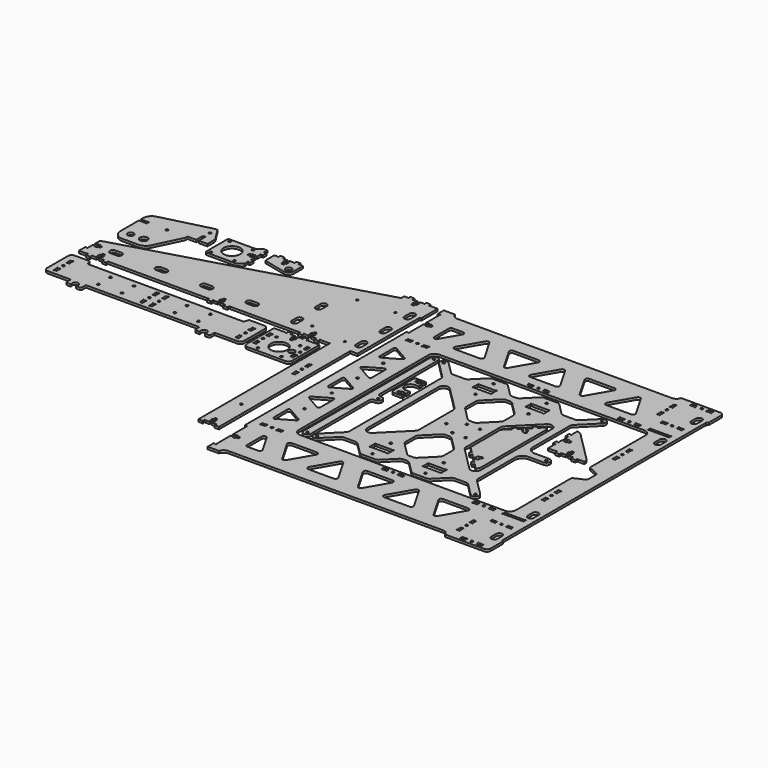
from build123d import *

# Parameters (mm, degrees)
F1_R      = 1.6
F1_R_2    = 11.1
F2_DEPTH  = 3
F1_R_3    = 4
F1_R_4    = 5
F3_DEPTH  = 3
F4_DEPTH  = 3
F5_DEPTH  = 3
F6_DEPTH  = 3
F1_R_5    = 1.3
F7_DEPTH  = 3
F8_DEPTH  = 3
F9_DEPTH  = 3
F10_DEPTH = 3
F11_DEPTH = 3
F12_DEPTH = 3
F13_DEPTH = 3


# Not quite as in the source:
# - ends of sketch curves that miss each other by under 0.0002 mm in the source are joined


with BuildPart() as f2:
    # F1 (on Top) → F2 (new body)
    with BuildSketch(Plane.XY):
        with BuildLine():
            Line((-94.274861, 295.883752), (-97.274861, 295.883752))
            Line((-97.274861, 295.883752), (-97.274861, 299.083764))
            Line((-97.274861, 299.083764), (-94.274861, 299.083764))
            Line((-94.274861, 299.083764), (-94.274861, 300.358758))
            Line((-94.274861, 300.358758), (-90.274833, 300.358758))
            Line((-90.274833, 300.358758), (-90.274833, 299.083764))
            Line((-90.274833, 299.083764), (-87.274861, 299.083764))
            Line((-87.274861, 299.083764), (-87.274861, 304.217735))
            ThreePointArc((-87.274861, 304.217735), (-87.3418483354, 304.4677350645), (-87.5248611291, 304.6507477764))
            ThreePointArc((-87.5248611291, 304.6507477764), (-87.628415003, 305.4373127782), (-86.8418493396, 305.3337618039))
            ThreePointArc((-86.8418493396, 305.3337618039), (-86.658837473, 305.1507499939), (-86.408838, 305.083763))
            Line((-86.408838, 305.083763), (-84.774809, 305.083763))
            ThreePointArc((-84.774809, 305.083763), (-84.4212556094, 305.2302096094), (-84.274809, 305.583763))
            Line((-84.274809, 305.583763), (-84.274809, 310.58376))
            ThreePointArc((-84.274809, 310.58376), (-84.4212556094, 310.9373133906), (-84.774809, 311.08376))
            Line((-84.774809, 311.08376), (-86.408836, 311.083757))
            ThreePointArc((-86.408836, 311.083757), (-86.6588360645, 311.0167696646), (-86.8418487764, 310.8337568709))
            ThreePointArc((-86.8418487764, 310.8337568709), (-87.6284139076, 310.7302031264), (-87.5248620539, 311.5167690934))
            ThreePointArc((-87.5248620539, 311.5167690934), (-87.3418506524, 311.6997821185), (-87.274864, 311.949781))
            Line((-87.274864, 311.949781), (-87.274861, 316.48375))
            Line((-87.274861, 316.48375), (-92.476156, 316.48375))
            ThreePointArc((-92.476156, 316.48375), (-92.7932522482, 316.4321433622), (-93.0776199539, 316.2826499388))
            Line((-93.0776199539, 316.2826499388), (-99.18468, 311.684851))
            ThreePointArc((-99.18468, 311.684851), (-99.4664969899, 311.5362133047), (-99.7807630779, 311.4837644773))
            ThreePointArc((-99.7807630779, 311.4837644773), (-99.7834535292, 311.4837536193), (-99.786144, 311.48375))
            Line((-99.786144, 311.48375), (-101.786144, 311.48375))
            Line((-101.786144, 311.48375), (-133.274827, 311.483751))
            ThreePointArc((-133.274827, 311.483751), (-134.6890405624, 310.8979645624), (-135.274827, 309.483751))
            Line((-135.274827, 309.483751), (-135.274827, 275.483767))
            ThreePointArc((-135.274827, 275.483767), (-134.6890405624, 274.0695534376), (-133.274827, 273.483767))
            Line((-133.274827, 273.483767), (-96.250499, 273.483766))
            Line((-96.250499, 273.483766), (-94.398561, 273.483766))
            Line((-94.398561, 273.483766), (-94.255412, 273.483766))
            Line((-94.255412, 273.483766), (-94.250499, 273.483766))
            ThreePointArc((-94.250499, 273.483766), (-94.250295, 273.4837660208), (-94.250091, 273.4837660832))
            ThreePointArc((-94.250091, 273.4837660832), (-93.933209001, 273.5354374406), (-93.6490345656, 273.684866423))
            Line((-93.6490345656, 273.684866423), (-87.274864, 278.483764))
            Line((-87.274864, 278.483764), (-87.274861, 283.017733))
            ThreePointArc((-87.274861, 283.017733), (-87.3418483354, 283.2677330645), (-87.5248611291, 283.4507457764))
            ThreePointArc((-87.5248611291, 283.4507457764), (-87.628415003, 284.2373117782), (-86.8418493396, 284.1337608039))
            ThreePointArc((-86.8418493396, 284.1337608039), (-86.658837473, 283.9507489939), (-86.408838, 283.883762))
            Line((-86.408838, 283.883762), (-84.774809, 283.883762))
            ThreePointArc((-84.774809, 283.883762), (-84.4212556094, 284.0302086094), (-84.274809, 284.383762))
            Line((-84.274809, 284.383762), (-84.274809, 289.383759))
            ThreePointArc((-84.274809, 289.383759), (-84.4212556094, 289.7373123906), (-84.774809, 289.883759))
            Line((-84.774809, 289.883759), (-86.408836, 289.883756))
            ThreePointArc((-86.408836, 289.883756), (-86.6588360645, 289.8167686646), (-86.8418487764, 289.6337558709))
            ThreePointArc((-86.8418487764, 289.6337558709), (-87.6284139076, 289.5302021264), (-87.5248620539, 290.3167680934))
            ThreePointArc((-87.5248620539, 290.3167680934), (-87.3418506524, 290.4997811185), (-87.274864, 290.74978))
            Line((-87.274864, 290.74978), (-87.274861, 295.883752))
            Line((-87.274861, 295.883752), (-90.274833, 295.883752))
            Line((-90.274833, 295.883752), (-90.274833, 294.608758))
            Line((-90.274833, 294.608758), (-94.274861, 294.608758))
            Line((-94.274861, 294.608758), (-94.274861, 295.883752))
        make_face()
        with Locations((-130.55856, 276.983762)):
            Circle(F1_R, mode=Mode.SUBTRACT)
        with Locations((-130.55856, 307.983762)):
            Circle(F1_R, mode=Mode.SUBTRACT)
        with Locations((-99.55856, 276.983762)):
            Circle(F1_R, mode=Mode.SUBTRACT)
        with Locations((-115.05856, 292.483762)):
            Circle(F1_R_2, mode=Mode.SUBTRACT)
        with Locations((-99.55856, 307.983762)):
            Circle(F1_R, mode=Mode.SUBTRACT)
    extrude(amount=F2_DEPTH)


with BuildPart() as f3:
    # F1 (on Top) → F3 (new body)
    with BuildSketch(Plane.XY):
        with BuildLine():
            Line((-159.410467, 320.207611), (-224.228619, 303.897463))
            ThreePointArc((-224.228619, 303.897463), (-230.4165571255, 299.5682679537), (-232.7929969991, 292.399932))
            Line((-232.7929969991, 292.399932), (-232.793028, 289.163531))
            Line((-232.793028, 289.163531), (-223.658684, 289.163423))
            ThreePointArc((-223.658684, 289.163423), (-223.4086688612, 289.2303497734), (-223.2256123858, 289.4133172229))
            ThreePointArc((-223.2256123858, 289.4133172229), (-222.4390222368, 289.5166799974), (-222.542765117, 288.7301392028))
            ThreePointArc((-222.542765117, 288.7301392028), (-222.7258213854, 288.5471694422), (-222.7928689854, 288.297186))
            Line((-222.7928689854, 288.297186), (-222.793243, 286.729319))
            ThreePointArc((-222.793243, 286.729319), (-222.7263163851, 286.4793031359), (-222.5433484605, 286.2962462029))
            ThreePointArc((-222.5433484605, 286.2962462029), (-222.4399864857, 285.509655754), (-223.2265267972, 285.613399117))
            ThreePointArc((-223.2265267972, 285.613399117), (-223.4094949908, 285.7964556355), (-223.659479, 285.8635029856))
            Line((-223.659479, 285.8635029856), (-232.793067, 285.863612))
            Line((-232.793067, 285.863612), (-232.793429, 255.338372))
            ThreePointArc((-232.793429, 255.338372), (-229.2788141866, 246.8530523388), (-220.793578, 243.3382350008))
            Line((-220.793578, 243.3382350008), (-199.185776, 243.337971))
            ThreePointArc((-199.185776, 243.337971), (-192.891904432, 245.1208782492), (-188.4683004288, 249.9399347123))
            Line((-188.4683004288, 249.9399347123), (-171.14421, 285.850619))
            Line((-171.14421, 285.850619), (-171.143584, 288.341917))
            ThreePointArc((-171.143584, 288.341917), (-171.2105107734, 288.5919321388), (-171.3934782229, 288.7749886142))
            ThreePointArc((-171.3934782229, 288.7749886142), (-171.4968409974, 289.5615787632), (-170.7103002028, 289.457835883))
            ThreePointArc((-170.7103002028, 289.457835883), (-170.5273304422, 289.2747796146), (-170.277347, 289.2077320146))
            Line((-170.277347, 289.2077320146), (-159.617928, 289.207691))
            Line((-159.617928, 289.207691), (-159.617812, 298.990524))
            ThreePointArc((-159.617812, 298.990524), (-159.6847389898, 299.2405395138), (-159.8677069727, 299.4235960473))
            ThreePointArc((-159.8677069727, 299.4235960473), (-159.9710686912, 300.2101870692), (-159.1845282028, 300.106443883))
            ThreePointArc((-159.1845282028, 300.106443883), (-159.0015590092, 299.9233873645), (-158.751575, 299.8563400144))
            Line((-158.751575, 299.8563400144), (-157.183708, 299.855966))
            ThreePointArc((-157.183708, 299.855966), (-156.9336924862, 299.9228929898), (-156.7506359527, 300.1058609727))
            ThreePointArc((-156.7506359527, 300.1058609727), (-155.9640452368, 300.2092229974), (-156.067788117, 299.4226822028))
            ThreePointArc((-156.067788117, 299.4226822028), (-156.2508446355, 299.2397130092), (-156.3178919856, 298.989729))
            Line((-156.3178919856, 298.989729), (-156.318008, 289.207652))
            Line((-156.318008, 289.207652), (-144.793374, 289.204907))
            Line((-144.793374, 289.204907), (-144.792923, 298.673118))
            ThreePointArc((-144.792923, 298.673118), (-145.0781392863, 301.2739997357), (-145.920290601, 303.7512391864))
            Line((-145.920290601, 303.7512391864), (-156.317603, 320.20762))
            Line((-156.317603, 320.20762), (-159.410467, 320.207611))
        make_face()
        with Locations((-220.093038, 256.71262)):
            Circle(F1_R_3, mode=Mode.SUBTRACT)
        with Locations((-203.093039, 256.708518)):
            Circle(F1_R_4, mode=Mode.SUBTRACT)
        with Locations((-196.968055, 287.512945)):
            Circle(F1_R, mode=Mode.SUBTRACT)
        with Locations((-157.968127, 309.857674)):
            Circle(F1_R, mode=Mode.SUBTRACT)
    extrude(amount=F3_DEPTH)


with BuildPart() as f4:
    # F1 (on Top) → F4 (new body)
    with BuildSketch(Plane.XY):
        with BuildLine():
            Line((506.328806, -37.510219), (506.328806, 298.489776))
            Line((506.328806, 298.489776), (508.328806, 300.48978))
            Line((508.328806, 300.48978), (508.328806, 320.489776))
            ThreePointArc((508.328806, 320.489776), (506.864340613, 324.0253121988), (503.328806, 325.489779))
            Line((503.328806, 325.489779), (451.978806, 325.489771))
            ThreePointArc((451.978806, 325.489771), (449.1318170616, 321.1652200468), (444.232839, 319.489777))
            Line((444.232839, 319.489777), (161.074772, 319.489774))
            ThreePointArc((161.074772, 319.489774), (156.1757937505, 321.1652176626), (153.3288040156, 325.489768004))
            Line((153.3288040156, 325.489768004), (138.328805, 325.489771))
            Line((138.328805, 325.489771), (138.328805, 315.489781))
            Line((138.328805, 315.489781), (140.562825, 315.489781))
            ThreePointArc((140.562825, 315.489781), (140.812824848, 315.5567682104), (140.9958375264, 315.7397806961))
            ThreePointArc((140.9958375264, 315.7397806961), (141.7824037309, 315.8433350503), (141.6788524869, 315.0567691566))
            ThreePointArc((141.6788524869, 315.0567691566), (141.4958407774, 314.873756098), (141.428854, 314.623757))
            Line((141.428854, 314.623757), (141.428851, 291.264785))
            Line((141.428851, 291.264785), (144.428822, 291.264785))
            Line((144.428822, 291.264785), (144.428822, 292.53978))
            Line((144.428822, 292.53978), (148.428851, 292.53978))
            Line((148.428851, 292.53978), (148.428851, 291.264785))
            Line((148.428851, 291.264785), (151.428851, 291.264785))
            Line((151.428851, 291.264785), (151.428851, 288.064774))
            Line((151.428851, 288.064774), (148.428851, 288.064774))
            Line((148.428851, 288.064774), (148.428851, 286.78978))
            Line((148.428851, 286.78978), (144.428822, 286.78978))
            Line((144.428822, 286.78978), (144.428822, 288.064774))
            Line((144.428822, 288.064774), (141.428851, 288.064774))
            Line((141.428851, 288.064774), (141.428851, 264.705804))
            ThreePointArc((141.428851, 264.705804), (141.4958382104, 264.455804152), (141.6788506961, 264.2727914736))
            ThreePointArc((141.6788506961, 264.2727914736), (141.7824048736, 263.4862250924), (140.9958389066, 263.5897769461))
            ThreePointArc((140.9958389066, 263.5897769461), (140.812826098, 263.7727882226), (140.562827, 263.839775))
            Line((140.562827, 263.839775), (138.328805, 263.839778))
            Line((138.328805, 263.839778), (138.328805, -2.860221))
            Line((138.328805, -2.860221), (140.562825, -2.860221))
            ThreePointArc((140.562825, -2.860221), (140.812824848, -2.7932337896), (140.9958375264, -2.6102213039))
            ThreePointArc((140.9958375264, -2.6102213039), (141.7824037309, -2.5066669497), (141.6788524869, -3.2932328434))
            ThreePointArc((141.6788524869, -3.2932328434), (141.4958407774, -3.476245902), (141.428854, -3.726245))
            Line((141.428854, -3.726245), (141.428851, -27.085217))
            Line((141.428851, -27.085217), (144.428822, -27.085217))
            Line((144.428822, -27.085217), (144.428822, -25.810223))
            Line((144.428822, -25.810223), (148.428851, -25.810223))
            Line((148.428851, -25.810223), (148.428851, -27.085217))
            Line((148.428851, -27.085217), (151.428851, -27.085217))
            Line((151.428851, -27.085217), (151.428851, -30.285228))
            Line((151.428851, -30.285228), (148.428851, -30.285228))
            Line((148.428851, -30.285228), (148.428851, -31.560223))
            Line((148.428851, -31.560223), (144.428822, -31.560223))
            Line((144.428822, -31.560223), (144.428822, -30.285228))
            Line((144.428822, -30.285228), (141.428851, -30.285228))
            Line((141.428851, -30.285228), (141.428851, -53.644198))
            ThreePointArc((141.428851, -53.644198), (141.4958382104, -53.894197848), (141.6788506961, -54.0772105264))
            ThreePointArc((141.6788506961, -54.0772105264), (141.7824048736, -54.8637769076), (140.9958389066, -54.7602250539))
            ThreePointArc((140.9958389066, -54.7602250539), (140.812826098, -54.5772137774), (140.562827, -54.510227))
            Line((140.562827, -54.510227), (138.328805, -54.510224))
            Line((138.328805, -54.510224), (138.328805, -64.510214))
            Line((138.328805, -64.510214), (153.328821, -64.510214))
            ThreePointArc((153.328821, -64.510214), (156.175804211, -60.1856730634), (161.074771, -58.510234))
            Line((161.074771, -58.510234), (444.23284, -58.510217))
            ThreePointArc((444.23284, -58.510217), (449.1318181012, -60.1856603223), (451.9788077731, -64.5102130586))
            Line((451.9788077731, -64.5102130586), (503.328806, -64.510214))
            ThreePointArc((503.328806, -64.510214), (506.8643360168, -63.0457488955), (508.328799, -59.510218))
            Line((508.328799, -59.510218), (508.328806, -39.510223))
            Line((508.328806, -39.510223), (506.328806, -37.510219))
        make_face()
        with BuildLine():
            ThreePointArc((167.66769, -12.134694), (169.8912328137, -9.2369165348), (173.2657661585, -10.6346939085))
            Line((173.2657661585, -10.6346939085), (186.966778, -34.365543))
            ThreePointArc((186.966778, -34.365543), (186.9667782378, -37.3655429542), (184.368702, -38.865543))
            Line((184.368702, -38.865543), (170.66769, -38.865543))
            ThreePointArc((170.66769, -38.865543), (168.5463696564, -37.9868633436), (167.66769, -35.865543))
            Line((167.66769, -35.865543), (167.66769, -12.134694))
        make_face(mode=Mode.SUBTRACT)
        with BuildLine():
            Line((200.965733, -3.938543), (234.367756, -3.938543))
            ThreePointArc((234.367756, -3.938543), (236.9658322378, -5.4385430458), (236.9658321585, -8.4385430915))
            Line((236.9658321585, -8.4385430915), (220.264821, -37.365543))
            ThreePointArc((220.264821, -37.365543), (217.666744, -38.865543), (215.0686678415, -37.3655430915))
            Line((215.0686678415, -37.3655430915), (198.367657, -8.438543))
            ThreePointArc((198.367657, -8.438543), (198.3676567622, -5.4385430458), (200.965733, -3.938543))
        make_face(mode=Mode.SUBTRACT)
        with BuildLine():
            ThreePointArc((286.9667781585, -34.3655429085), (286.9667782378, -37.3655429542), (284.368702, -38.865543))
            Line((284.368702, -38.865543), (250.966679, -38.865543))
            ThreePointArc((250.966679, -38.865543), (248.3686027622, -37.3655429542), (248.3686028415, -34.3655429085))
            Line((248.3686028415, -34.3655429085), (265.069614, -5.438543))
            ThreePointArc((265.069614, -5.438543), (267.66769, -3.938543), (270.2657661585, -5.4385429085))
            Line((270.2657661585, -5.4385429085), (286.9667781585, -34.3655429085))
        make_face(mode=Mode.SUBTRACT)
        with BuildLine():
            Line((300.965733, -3.938543), (334.367756, -3.938543))
            ThreePointArc((334.367756, -3.938543), (336.9658322378, -5.4385430458), (336.9658321585, -8.4385430915))
            Line((336.9658321585, -8.4385430915), (320.264821, -37.365543))
            ThreePointArc((320.264821, -37.365543), (317.666744, -38.865543), (315.0686678415, -37.3655430915))
            Line((315.0686678415, -37.3655430915), (298.367657, -8.438543))
            ThreePointArc((298.367657, -8.438543), (298.3676567622, -5.4385430458), (300.965733, -3.938543))
        make_face(mode=Mode.SUBTRACT)
        with BuildLine():
            ThreePointArc((386.9667781585, -34.3655429085), (386.9667782378, -37.3655429542), (384.368702, -38.865543))
            Line((384.368702, -38.865543), (350.966679, -38.865543))
            ThreePointArc((350.966679, -38.865543), (348.3686027622, -37.3655429542), (348.3686028415, -34.3655429085))
            Line((348.3686028415, -34.3655429085), (365.069614, -5.438543))
            ThreePointArc((365.069614, -5.438543), (367.66769, -3.938543), (370.2657661585, -5.4385429085))
            Line((370.2657661585, -5.4385429085), (386.9667781585, -34.3655429085))
        make_face(mode=Mode.SUBTRACT)
        with BuildLine():
            Line((469.628804, -60.114154), (469.628807, -58.546287))
            ThreePointArc((469.628807, -58.546287), (469.5618196646, -58.2962869355), (469.3788068709, -58.1132742236))
            ThreePointArc((469.3788068709, -58.1132742236), (469.275252997, -57.3267082218), (470.0618186604, -57.4302591961))
            ThreePointArc((470.0618186604, -57.4302591961), (470.244830527, -57.6132710061), (470.49483, -57.680258))
            Line((470.49483, -57.680258), (474.96278, -57.680258))
            ThreePointArc((474.96278, -57.680258), (475.212779848, -57.6132707896), (475.3957925264, -57.4302583039))
            ThreePointArc((475.3957925264, -57.4302583039), (476.1823577309, -57.3267039497), (476.0788064869, -58.1132698434))
            ThreePointArc((476.0788064869, -58.1132698434), (475.8957947774, -58.296282902), (475.828808, -58.546282))
            Line((475.828808, -58.546282), (475.828805, -60.114152))
            ThreePointArc((475.828805, -60.114152), (475.8957922104, -60.364151848), (476.0788046961, -60.5471645264))
            ThreePointArc((476.0788046961, -60.5471645264), (476.1823588736, -61.3337309076), (475.3957929066, -61.2301790539))
            ThreePointArc((475.3957929066, -61.2301790539), (475.212781098, -61.0471677774), (474.962782, -60.980181))
            Line((474.962782, -60.980181), (470.494832, -60.980178))
            ThreePointArc((470.494832, -60.980178), (470.2448319355, -61.0471653354), (470.0618192236, -61.2301781291))
            ThreePointArc((470.0618192236, -61.2301781291), (469.2752542218, -61.333732003), (469.3788051961, -60.5471663396))
            ThreePointArc((469.3788051961, -60.5471663396), (469.5618171311, -60.3641532565), (469.628804, -60.114154))
        make_face(mode=Mode.SUBTRACT)
        with BuildLine():
            Line((457.467739, -48.51023), (455.899872, -48.510227))
            ThreePointArc((455.899872, -48.510227), (455.6498719355, -48.5772143354), (455.4668592236, -48.7602271291))
            ThreePointArc((455.4668592236, -48.7602271291), (454.6802942218, -48.863781003), (454.7838451961, -48.0772153396))
            ThreePointArc((454.7838451961, -48.0772153396), (454.9668571311, -47.8942022565), (455.033844, -47.644203))
            Line((455.033844, -47.644203), (455.033844, -43.176253))
            ThreePointArc((455.033844, -43.176253), (454.9668566646, -42.9262529355), (454.7838438709, -42.7432402236))
            ThreePointArc((454.7838438709, -42.7432402236), (454.680289997, -41.9566752218), (455.4668556604, -42.0602261961))
            ThreePointArc((455.4668556604, -42.0602261961), (455.649867527, -42.2432380061), (455.899867, -42.310225))
            Line((455.899867, -42.310225), (457.467738, -42.310228))
            ThreePointArc((457.467738, -42.310228), (457.717737848, -42.2432407896), (457.9007505264, -42.0602283039))
            ThreePointArc((457.9007505264, -42.0602283039), (458.6873157309, -41.9566739497), (458.5837644869, -42.7432398434))
            ThreePointArc((458.5837644869, -42.7432398434), (458.4007527774, -42.926251902), (458.333766, -43.176251))
            Line((458.333766, -43.176251), (458.333763, -47.644201))
            ThreePointArc((458.333763, -47.644201), (458.4007502104, -47.894200848), (458.5837626961, -48.0772135264))
            ThreePointArc((458.5837626961, -48.0772135264), (458.6873168736, -48.8637799076), (457.9007509066, -48.7602280539))
            ThreePointArc((457.9007509066, -48.7602280539), (457.717738098, -48.5772167774), (457.467739, -48.51023))
        make_face(mode=Mode.SUBTRACT)
        with Locations((483.328806, -59.33022)):
            Circle(F1_R, mode=Mode.SUBTRACT)
        with BuildLine():
            Line((490.828803, -60.114154), (490.828806, -58.546287))
            ThreePointArc((490.828806, -58.546287), (490.7618186646, -58.2962869355), (490.5788058709, -58.1132742236))
            ThreePointArc((490.5788058709, -58.1132742236), (490.475251997, -57.3267082218), (491.2618176604, -57.4302591961))
            ThreePointArc((491.2618176604, -57.4302591961), (491.444830527, -57.6132710061), (491.69483, -57.680258))
            Line((491.69483, -57.680258), (496.162779, -57.680258))
            ThreePointArc((496.162779, -57.680258), (496.412778848, -57.6132707896), (496.5957915264, -57.4302583039))
            ThreePointArc((496.5957915264, -57.4302583039), (497.3823577309, -57.3267039497), (497.2788064869, -58.1132698434))
            ThreePointArc((497.2788064869, -58.1132698434), (497.0957947774, -58.296282902), (497.028808, -58.546282))
            Line((497.028808, -58.546282), (497.028805, -60.114152))
            ThreePointArc((497.028805, -60.114152), (497.0957922104, -60.364151848), (497.2788046961, -60.5471645264))
            ThreePointArc((497.2788046961, -60.5471645264), (497.3823588736, -61.3337309076), (496.5957929066, -61.2301790539))
            ThreePointArc((496.5957929066, -61.2301790539), (496.412780098, -61.0471677774), (496.162781, -60.980181))
            Line((496.162781, -60.980181), (491.694831, -60.980178))
            ThreePointArc((491.694831, -60.980178), (491.4448309355, -61.0471653354), (491.2618182236, -61.2301781291))
            ThreePointArc((491.2618182236, -61.2301781291), (490.4752532218, -61.333732003), (490.5788041961, -60.5471663396))
            ThreePointArc((490.5788041961, -60.5471663396), (490.7618161311, -60.3641532565), (490.828803, -60.114154))
        make_face(mode=Mode.SUBTRACT)
        with BuildLine():
            Line((400.965733, -3.938543), (434.367756, -3.938543))
            ThreePointArc((434.367756, -3.938543), (436.9658322378, -5.4385430458), (436.9658321585, -8.4385430915))
            Line((436.9658321585, -8.4385430915), (420.264821, -37.365543))
            ThreePointArc((420.264821, -37.365543), (417.666744, -38.865543), (415.0686678415, -37.3655430915))
            Line((415.0686678415, -37.3655430915), (398.367657, -8.438543))
            ThreePointArc((398.367657, -8.438543), (398.3676567622, -5.4385430458), (400.965733, -3.938543))
        make_face(mode=Mode.SUBTRACT)
        with Locations((456.683805, -34.810227)):
            Circle(F1_R, mode=Mode.SUBTRACT)
        with BuildLine():
            Line((457.467739, -27.31023), (455.899872, -27.310227))
            ThreePointArc((455.899872, -27.310227), (455.6498719355, -27.3772143354), (455.4668592236, -27.5602271291))
            ThreePointArc((455.4668592236, -27.5602271291), (454.6802942218, -27.663781003), (454.7838451961, -26.8772153396))
            ThreePointArc((454.7838451961, -26.8772153396), (454.9668571311, -26.6942032565), (455.033844, -26.444204))
            Line((455.033844, -26.444204), (455.033844, -21.976254))
            ThreePointArc((455.033844, -21.976254), (454.9668566646, -21.7262539355), (454.7838438709, -21.5432412236))
            ThreePointArc((454.7838438709, -21.5432412236), (454.680289997, -20.7566752218), (455.4668556604, -20.8602261961))
            ThreePointArc((455.4668556604, -20.8602261961), (455.649867527, -21.0432380061), (455.899867, -21.110225))
            Line((455.899867, -21.110225), (457.467738, -21.110228))
            ThreePointArc((457.467738, -21.110228), (457.717737848, -21.0432407896), (457.9007505264, -20.8602283039))
            ThreePointArc((457.9007505264, -20.8602283039), (458.6873157309, -20.7566739497), (458.5837644869, -21.5432398434))
            ThreePointArc((458.5837644869, -21.5432398434), (458.4007527774, -21.726252902), (458.333766, -21.976252))
            Line((458.333766, -21.976252), (458.333763, -26.444202))
            ThreePointArc((458.333763, -26.444202), (458.4007502104, -26.694201848), (458.5837626961, -26.8772145264))
            ThreePointArc((458.5837626961, -26.8772145264), (458.6873168736, -27.6637799076), (457.9007509066, -27.5602280539))
            ThreePointArc((457.9007509066, -27.5602280539), (457.717738098, -27.3772167774), (457.467739, -27.31023))
        make_face(mode=Mode.SUBTRACT)
        with BuildLine():
            Line((500.328806, -30.51022), (500.328806, -38.510221))
            ThreePointArc((500.328806, -38.510221), (496.328806, -42.510221), (492.328806, -38.51022))
            Line((492.328806, -38.51022), (492.328805, -30.51022))
            ThreePointArc((492.328805, -30.51022), (496.328806, -26.510221), (500.328806, -30.51022))
        make_face(mode=Mode.SUBTRACT)
        with BuildLine():
            Line((469.628804, -11.074154), (469.628807, -9.506287))
            ThreePointArc((469.628807, -9.506287), (469.5618196646, -9.2562869355), (469.3788068709, -9.0732742236))
            ThreePointArc((469.3788068709, -9.0732742236), (469.275252997, -8.2867082218), (470.0618186604, -8.3902591961))
            ThreePointArc((470.0618186604, -8.3902591961), (470.244830527, -8.5732710061), (470.49483, -8.640258))
            Line((470.49483, -8.640258), (474.96278, -8.640258))
            ThreePointArc((474.96278, -8.640258), (475.212779848, -8.5732707896), (475.3957925264, -8.3902583039))
            ThreePointArc((475.3957925264, -8.3902583039), (476.1823577309, -8.2867039497), (476.0788064869, -9.0732698434))
            ThreePointArc((476.0788064869, -9.0732698434), (475.8957947774, -9.256282902), (475.828808, -9.506282))
            Line((475.828808, -9.506282), (475.828805, -11.074152))
            ThreePointArc((475.828805, -11.074152), (475.8957922104, -11.324151848), (476.0788046961, -11.5071645264))
            ThreePointArc((476.0788046961, -11.5071645264), (476.1823588736, -12.2937309076), (475.3957929066, -12.1901790539))
            ThreePointArc((475.3957929066, -12.1901790539), (475.212781098, -12.0071677774), (474.962782, -11.940181))
            Line((474.962782, -11.940181), (470.494832, -11.940178))
            ThreePointArc((470.494832, -11.940178), (470.2448319355, -12.0071653354), (470.0618192236, -12.1901781291))
            ThreePointArc((470.0618192236, -12.1901781291), (469.2752542218, -12.293732003), (469.3788051961, -11.5071663396))
            ThreePointArc((469.3788051961, -11.5071663396), (469.5618171311, -11.3241532565), (469.628804, -11.074154))
        make_face(mode=Mode.SUBTRACT)
        with Locations((483.328806, -10.290219)):
            Circle(F1_R, mode=Mode.SUBTRACT)
        with BuildLine():
            Line((490.828803, -11.074154), (490.828806, -9.506287))
            ThreePointArc((490.828806, -9.506287), (490.7618186646, -9.2562869355), (490.5788058709, -9.0732742236))
            ThreePointArc((490.5788058709, -9.0732742236), (490.475251997, -8.2867082218), (491.2618176604, -8.3902591961))
            ThreePointArc((491.2618176604, -8.3902591961), (491.444830527, -8.5732710061), (491.69483, -8.640258))
            Line((491.69483, -8.640258), (496.162779, -8.640258))
            ThreePointArc((496.162779, -8.640258), (496.412778848, -8.5732707896), (496.5957915264, -8.3902583039))
            ThreePointArc((496.5957915264, -8.3902583039), (497.3823577309, -8.2867039497), (497.2788064869, -9.0732698434))
            ThreePointArc((497.2788064869, -9.0732698434), (497.0957947774, -9.256282902), (497.028808, -9.506282))
            Line((497.028808, -9.506282), (497.028805, -11.074152))
            ThreePointArc((497.028805, -11.074152), (497.0957922104, -11.324151848), (497.2788046961, -11.5071645264))
            ThreePointArc((497.2788046961, -11.5071645264), (497.3823588736, -12.2937309076), (496.5957929066, -12.1901790539))
            ThreePointArc((496.5957929066, -12.1901790539), (496.412780098, -12.0071677774), (496.162781, -11.940181))
            Line((496.162781, -11.940181), (491.694831, -11.940178))
            ThreePointArc((491.694831, -11.940178), (491.4448309355, -12.0071653354), (491.2618182236, -12.1901781291))
            ThreePointArc((491.2618182236, -12.1901781291), (490.4752532218, -12.293732003), (490.5788041961, -11.5071663396))
            ThreePointArc((490.5788041961, -11.5071663396), (490.7618161311, -11.3241532565), (490.828803, -11.074154))
        make_face(mode=Mode.SUBTRACT)
        with BuildLine():
            Line((149.6288, 9.530845), (149.628803, 11.098712))
            ThreePointArc((149.628803, 11.098712), (149.5618156646, 11.3487120645), (149.3788028709, 11.5317247764))
            ThreePointArc((149.3788028709, 11.5317247764), (149.275248997, 12.3182897782), (150.0618146604, 12.2147388039))
            ThreePointArc((150.0618146604, 12.2147388039), (150.244826527, 12.0317269939), (150.494826, 11.96474))
            Line((150.494826, 11.96474), (154.962776, 11.96474))
            ThreePointArc((154.962776, 11.96474), (155.212775848, 12.0317272104), (155.3957885264, 12.2147396961))
            ThreePointArc((155.3957885264, 12.2147396961), (156.1823537309, 12.3182940503), (156.0788024869, 11.5317281566))
            ThreePointArc((156.0788024869, 11.5317281566), (155.8957907774, 11.348716098), (155.828804, 11.098717))
            Line((155.828804, 11.098717), (155.828801, 9.530846))
            ThreePointArc((155.828801, 9.530846), (155.8957882104, 9.280846152), (156.0788006961, 9.0978334736))
            ThreePointArc((156.0788006961, 9.0978334736), (156.1823548736, 8.3112680924), (155.3957889066, 8.4148199461))
            ThreePointArc((155.3957889066, 8.4148199461), (155.212777098, 8.5978312226), (154.962778, 8.664818))
            Line((154.962778, 8.664818), (150.494828, 8.664821))
            ThreePointArc((150.494828, 8.664821), (150.2448279355, 8.5978336646), (150.0618152236, 8.4148208709))
            ThreePointArc((150.0618152236, 8.4148208709), (149.2752502218, 8.311266997), (149.3788011961, 9.0978326604))
            ThreePointArc((149.3788011961, 9.0978326604), (149.5618131311, 9.2808457435), (149.6288, 9.530845))
        make_face(mode=Mode.SUBTRACT)
        with Locations((163.328802, 10.314779)):
            Circle(F1_R, mode=Mode.SUBTRACT)
        with BuildLine():
            Line((170.828799, 9.530845), (170.828802, 11.098712))
            ThreePointArc((170.828802, 11.098712), (170.7618146646, 11.3487120645), (170.5788018709, 11.5317247764))
            ThreePointArc((170.5788018709, 11.5317247764), (170.475247997, 12.3182897782), (171.2618136604, 12.2147388039))
            ThreePointArc((171.2618136604, 12.2147388039), (171.444826527, 12.0317269939), (171.694826, 11.96474))
            Line((171.694826, 11.96474), (176.162775, 11.96474))
            ThreePointArc((176.162775, 11.96474), (176.412774848, 12.0317272104), (176.5957875264, 12.2147396961))
            ThreePointArc((176.5957875264, 12.2147396961), (177.3823537309, 12.3182940503), (177.2788024869, 11.5317281566))
            ThreePointArc((177.2788024869, 11.5317281566), (177.0957907774, 11.348716098), (177.028804, 11.098717))
            Line((177.028804, 11.098717), (177.028801, 9.530846))
            ThreePointArc((177.028801, 9.530846), (177.0957882104, 9.280846152), (177.2788006961, 9.0978334736))
            ThreePointArc((177.2788006961, 9.0978334736), (177.3823548736, 8.3112680924), (176.5957889066, 8.4148199461))
            ThreePointArc((176.5957889066, 8.4148199461), (176.412776098, 8.5978312226), (176.162777, 8.664818))
            Line((176.162777, 8.664818), (171.694827, 8.664821))
            ThreePointArc((171.694827, 8.664821), (171.4448269355, 8.5978336646), (171.2618142236, 8.4148208709))
            ThreePointArc((171.2618142236, 8.4148208709), (170.4752492218, 8.311266997), (170.5788001961, 9.0978326604))
            ThreePointArc((170.5788001961, 9.0978326604), (170.7618121311, 9.2808457435), (170.828799, 9.530845))
        make_face(mode=Mode.SUBTRACT)
        with BuildLine():
            Line((150.636191, 29.161643), (150.636191, 51.708009))
            ThreePointArc((150.636191, 51.708009), (151.6486908793, 53.461710373), (153.6736907587, 53.461710582))
            Line((153.6736907587, 53.461710582), (173.199416, 42.188528))
            ThreePointArc((173.199416, 42.188528), (174.211916, 40.43482625), (173.1994161917, 38.681124668))
            Line((173.1994161917, 38.681124668), (153.673691, 27.407942))
            ThreePointArc((153.673691, 27.407942), (151.6486910958, 27.407941502), (150.636191, 29.161643))
        make_face(mode=Mode.SUBTRACT)
        with Locations((163.328802, 64.208019)):
            Circle(F1_R, mode=Mode.SUBTRACT)
        with BuildLine():
            ThreePointArc((171.1744162413, 101.008094582), (173.1994161207, 101.008094373), (174.211916, 99.254393))
            Line((174.211916, 99.254393), (174.211916, 76.708028))
            ThreePointArc((174.211916, 76.708028), (173.1994159042, 74.954326502), (171.1744158083, 74.954326668))
            Line((171.1744158083, 74.954326668), (151.648691, 86.227509))
            ThreePointArc((151.648691, 86.227509), (150.636191, 87.98121025), (151.6486912413, 89.734911582))
            Line((151.6486912413, 89.734911582), (171.1744162413, 101.008094582))
        make_face(mode=Mode.SUBTRACT)
        with Locations((163.328802, 109.231201)):
            Circle(F1_R, mode=Mode.SUBTRACT)
        with BuildLine():
            Line((150.636191, 119.208009), (150.636191, 141.754374))
            ThreePointArc((150.636191, 141.754374), (151.6486908793, 143.508075373), (153.6736907587, 143.508075582))
            Line((153.6736907587, 143.508075582), (173.199416, 132.234893))
            ThreePointArc((173.199416, 132.234893), (174.211916, 130.48119125), (173.1994161917, 128.727489668))
            Line((173.1994161917, 128.727489668), (153.673691, 117.454307))
            ThreePointArc((153.673691, 117.454307), (151.6486910958, 117.454307502), (150.636191, 119.208009))
        make_face(mode=Mode.SUBTRACT)
        with Locations((163.328802, 151.735476)):
            Circle(F1_R, mode=Mode.SUBTRACT)
        with BuildLine():
            Line((309.628796, 9.530845), (309.628799, 11.098712))
            ThreePointArc((309.628799, 11.098712), (309.5618116646, 11.3487120645), (309.3787988709, 11.5317247764))
            ThreePointArc((309.3787988709, 11.5317247764), (309.275244997, 12.3182897782), (310.0618106604, 12.2147388039))
            ThreePointArc((310.0618106604, 12.2147388039), (310.244823527, 12.0317269939), (310.494823, 11.96474))
            Line((310.494823, 11.96474), (314.962772, 11.96474))
            ThreePointArc((314.962772, 11.96474), (315.212771848, 12.0317272104), (315.3957845264, 12.2147396961))
            ThreePointArc((315.3957845264, 12.2147396961), (316.1823507309, 12.3182940503), (316.0787994869, 11.5317281566))
            ThreePointArc((316.0787994869, 11.5317281566), (315.8957877774, 11.348716098), (315.828801, 11.098717))
            Line((315.828801, 11.098717), (315.828798, 9.530846))
            ThreePointArc((315.828798, 9.530846), (315.8957852104, 9.280846152), (316.0787976961, 9.0978334736))
            ThreePointArc((316.0787976961, 9.0978334736), (316.1823518736, 8.3112680924), (315.3957859066, 8.4148199461))
            ThreePointArc((315.3957859066, 8.4148199461), (315.212773098, 8.5978312226), (314.962774, 8.664818))
            Line((314.962774, 8.664818), (310.494824, 8.664821))
            ThreePointArc((310.494824, 8.664821), (310.2448239355, 8.5978336646), (310.0618112236, 8.4148208709))
            ThreePointArc((310.0618112236, 8.4148208709), (309.2752462218, 8.311266997), (309.3787971961, 9.0978326604))
            ThreePointArc((309.3787971961, 9.0978326604), (309.5618091311, 9.2808457435), (309.628796, 9.530845))
        make_face(mode=Mode.SUBTRACT)
        with Locations((323.328798, 10.314779)):
            Circle(F1_R, mode=Mode.SUBTRACT)
        with BuildLine():
            Line((330.828795, 9.530845), (330.828798, 11.098712))
            ThreePointArc((330.828798, 11.098712), (330.7618106646, 11.3487120645), (330.5787978709, 11.5317247764))
            ThreePointArc((330.5787978709, 11.5317247764), (330.475243997, 12.3182897782), (331.2618096604, 12.2147388039))
            ThreePointArc((331.2618096604, 12.2147388039), (331.444822527, 12.0317269939), (331.694822, 11.96474))
            Line((331.694822, 11.96474), (336.162772, 11.96474))
            ThreePointArc((336.162772, 11.96474), (336.412771848, 12.0317272104), (336.5957845264, 12.2147396961))
            ThreePointArc((336.5957845264, 12.2147396961), (337.3823497309, 12.3182940503), (337.2787984869, 11.5317281566))
            ThreePointArc((337.2787984869, 11.5317281566), (337.0957867774, 11.348716098), (337.0288, 11.098717))
            Line((337.0288, 11.098717), (337.028797, 9.530846))
            ThreePointArc((337.028797, 9.530846), (337.0957842104, 9.280846152), (337.2787966961, 9.0978334736))
            ThreePointArc((337.2787966961, 9.0978334736), (337.3823508736, 8.3112680924), (336.5957849066, 8.4148199461))
            ThreePointArc((336.5957849066, 8.4148199461), (336.412773098, 8.5978312226), (336.162774, 8.664818))
            Line((336.162774, 8.664818), (331.694824, 8.664821))
            ThreePointArc((331.694824, 8.664821), (331.4448239355, 8.5978336646), (331.2618112236, 8.4148208709))
            ThreePointArc((331.2618112236, 8.4148208709), (330.4752452218, 8.311266997), (330.5787961961, 9.0978326604))
            ThreePointArc((330.5787961961, 9.0978326604), (330.7618081311, 9.2808457435), (330.828795, 9.530845))
        make_face(mode=Mode.SUBTRACT)
        with BuildLine():
            ThreePointArc((430.0617510934, 8.4148639461), (429.2751851264, 8.3113120924), (429.3787391291, 9.0978777764))
            ThreePointArc((429.3787391291, 9.0978777764), (429.5617517896, 9.280890152), (429.628739, 9.53089))
            Line((429.628739, 9.53089), (429.628736, 11.098758))
            ThreePointArc((429.628736, 11.098758), (429.5617490061, 11.348757473), (429.3787370539, 11.5317700934))
            ThreePointArc((429.3787370539, 11.5317700934), (429.2751863986, 12.3183351797), (430.0617515264, 12.2147813039))
            ThreePointArc((430.0617515264, 12.2147813039), (430.2447639355, 12.0317683354), (430.494764, 11.964781))
            Line((430.494764, 11.964781), (434.962714, 11.964784))
            ThreePointArc((434.962714, 11.964784), (435.212713473, 12.0317709939), (435.3957260934, 12.2147829461))
            ThreePointArc((435.3957260934, 12.2147829461), (436.182292003, 12.3183337782), (436.0787383039, 11.5317684736))
            ThreePointArc((436.0787383039, 11.5317684736), (435.8957253354, 11.3487560645), (435.828738, 11.098756))
            Line((435.828738, 11.098756), (435.828741, 9.530886))
            ThreePointArc((435.828741, 9.530886), (435.8957276524, 9.2808871185), (436.0787387631, 9.0978745896))
            ThreePointArc((436.0787387631, 9.0978745896), (436.1822909076, 8.3113081264), (435.3957252236, 8.4148621291))
            ThreePointArc((435.3957252236, 8.4148621291), (435.212711848, 8.5978747896), (434.962712, 8.664862))
            Line((434.962712, 8.664862), (430.494763, 8.664862))
            ThreePointArc((430.494763, 8.664862), (430.244763902, 8.5978752226), (430.0617510934, 8.4148639461))
        make_face(mode=Mode.SUBTRACT)
        with Locations((443.328738, 10.314823)):
            Circle(F1_R, mode=Mode.SUBTRACT)
        with BuildLine():
            ThreePointArc((451.2617500934, 8.4148639461), (450.4751841264, 8.3113120924), (450.5787381291, 9.0978777764))
            ThreePointArc((450.5787381291, 9.0978777764), (450.7617507896, 9.280890152), (450.828738, 9.53089))
            Line((450.828738, 9.53089), (450.828735, 11.098758))
            ThreePointArc((450.828735, 11.098758), (450.7617480061, 11.348757473), (450.5787360539, 11.5317700934))
            ThreePointArc((450.5787360539, 11.5317700934), (450.4751853986, 12.3183351797), (451.2617505264, 12.2147813039))
            ThreePointArc((451.2617505264, 12.2147813039), (451.4447639355, 12.0317683354), (451.694764, 11.964781))
            Line((451.694764, 11.964781), (456.162714, 11.964784))
            ThreePointArc((456.162714, 11.964784), (456.412713473, 12.0317709939), (456.5957260934, 12.2147829461))
            ThreePointArc((456.5957260934, 12.2147829461), (457.382291003, 12.3183337782), (457.2787373039, 11.5317684736))
            ThreePointArc((457.2787373039, 11.5317684736), (457.0957243354, 11.3487560645), (457.028737, 11.098756))
            Line((457.028737, 11.098756), (457.02874, 9.530886))
            ThreePointArc((457.02874, 9.530886), (457.0957266524, 9.2808871185), (457.2787377631, 9.0978745896))
            ThreePointArc((457.2787377631, 9.0978745896), (457.3822899076, 8.3113081264), (456.5957242236, 8.4148621291))
            ThreePointArc((456.5957242236, 8.4148621291), (456.412711848, 8.5978747896), (456.162712, 8.664862))
            Line((456.162712, 8.664862), (451.694762, 8.664862))
            ThreePointArc((451.694762, 8.664862), (451.444762902, 8.5978752226), (451.2617500934, 8.4148639461))
        make_face(mode=Mode.SUBTRACT)
        with BuildLine():
            Line((469.628804, 9.530845), (469.628807, 11.098712))
            ThreePointArc((469.628807, 11.098712), (469.5618196646, 11.3487120645), (469.3788068709, 11.5317247764))
            ThreePointArc((469.3788068709, 11.5317247764), (469.275252997, 12.3182897782), (470.0618186604, 12.2147388039))
            ThreePointArc((470.0618186604, 12.2147388039), (470.244830527, 12.0317269939), (470.49483, 11.96474))
            Line((470.49483, 11.96474), (496.162779, 11.96474))
            ThreePointArc((496.162779, 11.96474), (496.412778848, 12.0317272104), (496.5957915264, 12.2147396961))
            ThreePointArc((496.5957915264, 12.2147396961), (497.3823577309, 12.3182940503), (497.2788064869, 11.5317281566))
            ThreePointArc((497.2788064869, 11.5317281566), (497.0957947774, 11.348716098), (497.028808, 11.098717))
            Line((497.028808, 11.098717), (497.028805, 9.530846))
            ThreePointArc((497.028805, 9.530846), (497.0957922104, 9.280846152), (497.2788046961, 9.0978334736))
            ThreePointArc((497.2788046961, 9.0978334736), (497.3823588736, 8.3112680924), (496.5957929066, 8.4148199461))
            ThreePointArc((496.5957929066, 8.4148199461), (496.412780098, 8.5978312226), (496.162781, 8.664818))
            Line((496.162781, 8.664818), (470.494832, 8.664821))
            ThreePointArc((470.494832, 8.664821), (470.2448319355, 8.5978336646), (470.0618192236, 8.4148208709))
            ThreePointArc((470.0618192236, 8.4148208709), (469.2752542218, 8.311266997), (469.3788051961, 9.0978326604))
            ThreePointArc((469.3788051961, 9.0978326604), (469.5618171311, 9.2808457435), (469.628804, 9.530845))
        make_face(mode=Mode.SUBTRACT)
        with BuildLine():
            Line((500.328806, 29.48978), (500.328806, 21.489779))
            ThreePointArc((500.328806, 21.489779), (496.328806, 17.489779), (492.328806, 21.48978))
            Line((492.328806, 21.48978), (492.328805, 29.48978))
            ThreePointArc((492.328805, 29.48978), (496.328806, 33.489779), (500.328806, 29.48978))
        make_face(mode=Mode.SUBTRACT)
        with BuildLine():
            Line((484.112738, 58.264736), (482.544871, 58.264739))
            ThreePointArc((482.544871, 58.264739), (482.294871152, 58.1977517896), (482.1118584736, 58.0147393039))
            ThreePointArc((482.1118584736, 58.0147393039), (481.3252930924, 57.9111851264), (481.4288449461, 58.6977510934))
            ThreePointArc((481.4288449461, 58.6977510934), (481.6118562226, 58.880763902), (481.678843, 59.130763))
            Line((481.678843, 59.130763), (481.678843, 63.598713))
            ThreePointArc((481.678843, 63.598713), (481.6118557896, 63.848712848), (481.4288433039, 64.0317255264))
            ThreePointArc((481.4288433039, 64.0317255264), (481.3252891264, 64.8182909076), (482.1118550934, 64.7147390539))
            ThreePointArc((482.1118550934, 64.7147390539), (482.294866902, 64.5317277774), (482.544866, 64.464741))
            Line((482.544866, 64.464741), (484.112737, 64.464738))
            ThreePointArc((484.112737, 64.464738), (484.3627370645, 64.5317253354), (484.5457497764, 64.7147381291))
            ThreePointArc((484.5457497764, 64.7147381291), (485.3323147782, 64.818292003), (485.2287638039, 64.0317263396))
            ThreePointArc((485.2287638039, 64.0317263396), (485.0457519939, 63.848714473), (484.978765, 63.598715))
            Line((484.978765, 63.598715), (484.978762, 59.130765))
            ThreePointArc((484.978762, 59.130765), (485.0457493354, 58.8807649355), (485.2287621291, 58.6977522236))
            ThreePointArc((485.2287621291, 58.6977522236), (485.332316003, 57.9111862218), (484.5457503396, 58.0147371961))
            ThreePointArc((484.5457503396, 58.0147371961), (484.362737473, 58.1977490061), (484.112738, 58.264736))
        make_face(mode=Mode.SUBTRACT)
        with Locations((483.328804, 71.964739)):
            Circle(F1_R, mode=Mode.SUBTRACT)
        with BuildLine():
            Line((490.328805, 137.215689), (490.328805, 123.772045))
            ThreePointArc((490.328805, 123.772045), (490.01248077, 122.692584069), (489.1635690984, 121.9545827858))
            Line((489.1635690984, 121.9545827858), (476.369588, 116.078278))
            ThreePointArc((476.369588, 116.078278), (475.5206772547, 115.3402769694), (475.204353, 114.260817))
            Line((475.204353, 114.260817), (475.204329, 23.489778))
            ThreePointArc((475.204329, 23.489778), (472.8679762347, 17.8397019028), (467.2235309999, 15.4897780448))
            Line((467.2235309999, 15.4897780448), (196.328803, 15.489776))
            ThreePointArc((196.328803, 15.489776), (190.671958468, 17.8329335893), (188.328817, 23.489779))
            Line((188.328817, 23.489779), (188.328817, 237.489779))
            ThreePointArc((188.328817, 237.489779), (190.6719496292, 243.1466339566), (196.328803, 245.489781))
            Line((196.328803, 245.489781), (467.223588, 245.489781))
            ThreePointArc((467.223588, 245.489781), (472.8680322347, 243.1398570972), (475.204385, 237.489781))
            Line((475.204385, 237.489781), (475.204361, 146.817174))
            ThreePointArc((475.204361, 146.817174), (475.5175584266, 145.7426046782), (476.3590589845, 145.0045879668))
            Line((476.3590589845, 145.0045879668), (489.174106, 139.028274))
            ThreePointArc((489.174106, 139.028274), (490.0156069478, 138.2902583039), (490.328805, 137.215689))
        make_face(mode=Mode.SUBTRACT)
        with BuildLine():
            Line((484.112738, 79.464736), (482.544871, 79.464739))
            ThreePointArc((482.544871, 79.464739), (482.294871152, 79.3977517896), (482.1118584736, 79.2147393039))
            ThreePointArc((482.1118584736, 79.2147393039), (481.3252930924, 79.1111851264), (481.4288449461, 79.8977510934))
            ThreePointArc((481.4288449461, 79.8977510934), (481.6118562226, 80.080762902), (481.678843, 80.330762))
            Line((481.678843, 80.330762), (481.678843, 84.798712))
            ThreePointArc((481.678843, 84.798712), (481.6118557896, 85.048711848), (481.4288433039, 85.2317245264))
            ThreePointArc((481.4288433039, 85.2317245264), (481.3252891264, 86.0182909076), (482.1118550934, 85.9147390539))
            ThreePointArc((482.1118550934, 85.9147390539), (482.294866902, 85.7317277774), (482.544866, 85.664741))
            Line((482.544866, 85.664741), (484.112737, 85.664738))
            ThreePointArc((484.112737, 85.664738), (484.3627370645, 85.7317253354), (484.5457497764, 85.9147381291))
            ThreePointArc((484.5457497764, 85.9147381291), (485.3323147782, 86.018292003), (485.2287638039, 85.2317263396))
            ThreePointArc((485.2287638039, 85.2317263396), (485.0457519939, 85.048713473), (484.978765, 84.798714))
            Line((484.978765, 84.798714), (484.978762, 80.330764))
            ThreePointArc((484.978762, 80.330764), (485.0457493354, 80.0807639355), (485.2287621291, 79.8977512236))
            ThreePointArc((485.2287621291, 79.8977512236), (485.332316003, 79.1111862218), (484.5457503396, 79.2147371961))
            ThreePointArc((484.5457503396, 79.2147371961), (484.362737473, 79.3977490061), (484.112738, 79.464736))
        make_face(mode=Mode.SUBTRACT)
        with BuildLine():
            ThreePointArc((171.1744162413, 186.016643582), (173.1994161207, 186.016643373), (174.211916, 184.262942))
            Line((174.211916, 184.262942), (174.211916, 161.716577))
            ThreePointArc((174.211916, 161.716577), (173.1994159042, 159.962875502), (171.1744158083, 159.962875668))
            Line((171.1744158083, 159.962875668), (151.648691, 171.236058))
            ThreePointArc((151.648691, 171.236058), (150.636191, 172.98975925), (151.6486912413, 174.743460582))
            Line((151.6486912413, 174.743460582), (171.1744162413, 186.016643582))
        make_face(mode=Mode.SUBTRACT)
        with Locations((163.328802, 194.23975)):
            Circle(F1_R, mode=Mode.SUBTRACT)
        with BuildLine():
            Line((150.636191, 204.216558), (150.636191, 226.762923))
            ThreePointArc((150.636191, 226.762923), (151.6486908793, 228.516624373), (153.6736907587, 228.516624582))
            Line((153.6736907587, 228.516624582), (173.199416, 217.243442))
            ThreePointArc((173.199416, 217.243442), (174.211916, 215.48974025), (173.1994161917, 213.736038668))
            Line((173.1994161917, 213.736038668), (153.673691, 202.462856))
            ThreePointArc((153.673691, 202.462856), (151.6486910958, 202.462856502), (150.636191, 204.216558))
        make_face(mode=Mode.SUBTRACT)
        with BuildLine():
            Line((149.6288, 249.880845), (149.628803, 251.448713))
            ThreePointArc((149.628803, 251.448713), (149.5618156646, 251.6987130645), (149.3788028709, 251.8817257764))
            ThreePointArc((149.3788028709, 251.8817257764), (149.275248997, 252.6682907782), (150.0618146604, 252.5647398039))
            ThreePointArc((150.0618146604, 252.5647398039), (150.244826527, 252.3817279939), (150.494826, 252.314741))
            Line((150.494826, 252.314741), (154.962776, 252.314741))
            ThreePointArc((154.962776, 252.314741), (155.212775848, 252.3817282104), (155.3957885264, 252.5647406961))
            ThreePointArc((155.3957885264, 252.5647406961), (156.1823537309, 252.6682950503), (156.0788024869, 251.8817291566))
            ThreePointArc((156.0788024869, 251.8817291566), (155.8957907774, 251.698716098), (155.828804, 251.448717))
            Line((155.828804, 251.448717), (155.828801, 249.880847))
            ThreePointArc((155.828801, 249.880847), (155.8957882104, 249.630847152), (156.0788006961, 249.4478344736))
            ThreePointArc((156.0788006961, 249.4478344736), (156.1823548736, 248.6612690924), (155.3957889066, 248.7648209461))
            ThreePointArc((155.3957889066, 248.7648209461), (155.212777098, 248.9478322226), (154.962778, 249.014819))
            Line((154.962778, 249.014819), (150.494828, 249.014822))
            ThreePointArc((150.494828, 249.014822), (150.2448279355, 248.9478346646), (150.0618152236, 248.7648218709))
            ThreePointArc((150.0618152236, 248.7648218709), (149.2752502218, 248.661267997), (149.3788011961, 249.4478336604))
            ThreePointArc((149.3788011961, 249.4478336604), (149.5618131311, 249.6308457435), (149.6288, 249.880845))
        make_face(mode=Mode.SUBTRACT)
        with Locations((163.328802, 250.66478)):
            Circle(F1_R, mode=Mode.SUBTRACT)
        with BuildLine():
            Line((170.828799, 249.880845), (170.828802, 251.448713))
            ThreePointArc((170.828802, 251.448713), (170.7618146646, 251.6987130645), (170.5788018709, 251.8817257764))
            ThreePointArc((170.5788018709, 251.8817257764), (170.475247997, 252.6682907782), (171.2618136604, 252.5647398039))
            ThreePointArc((171.2618136604, 252.5647398039), (171.444826527, 252.3817279939), (171.694826, 252.314741))
            Line((171.694826, 252.314741), (176.162775, 252.314741))
            ThreePointArc((176.162775, 252.314741), (176.412774848, 252.3817282104), (176.5957875264, 252.5647406961))
            ThreePointArc((176.5957875264, 252.5647406961), (177.3823537309, 252.6682950503), (177.2788024869, 251.8817291566))
            ThreePointArc((177.2788024869, 251.8817291566), (177.0957907774, 251.698716098), (177.028804, 251.448717))
            Line((177.028804, 251.448717), (177.028801, 249.880847))
            ThreePointArc((177.028801, 249.880847), (177.0957882104, 249.630847152), (177.2788006961, 249.4478344736))
            ThreePointArc((177.2788006961, 249.4478344736), (177.3823548736, 248.6612690924), (176.5957889066, 248.7648209461))
            ThreePointArc((176.5957889066, 248.7648209461), (176.412776098, 248.9478322226), (176.162777, 249.014819))
            Line((176.162777, 249.014819), (171.694827, 249.014822))
            ThreePointArc((171.694827, 249.014822), (171.4448269355, 248.9478346646), (171.2618142236, 248.7648218709))
            ThreePointArc((171.2618142236, 248.7648218709), (170.4752492218, 248.661267997), (170.5788001961, 249.4478336604))
            ThreePointArc((170.5788001961, 249.4478336604), (170.7618121311, 249.6308457435), (170.828799, 249.880845))
        make_face(mode=Mode.SUBTRACT)
        with BuildLine():
            Line((186.966778, 295.3451), (173.265766, 271.614252))
            ThreePointArc((173.265766, 271.614252), (169.8912328137, 270.2164745348), (167.66769, 273.114252))
            Line((167.66769, 273.114252), (167.66769, 296.8451))
            ThreePointArc((167.66769, 296.8451), (168.5463696564, 298.9664203436), (170.66769, 299.8451))
            Line((170.66769, 299.8451), (184.368702, 299.8451))
            ThreePointArc((184.368702, 299.8451), (186.9667782378, 298.3450999542), (186.966778, 295.3451))
        make_face(mode=Mode.SUBTRACT)
        with BuildLine():
            ThreePointArc((236.9658321585, 269.4181000915), (236.9658322378, 266.4181000458), (234.367756, 264.9181))
            Line((234.367756, 264.9181), (200.965733, 264.9181))
            ThreePointArc((200.965733, 264.9181), (198.3676567622, 266.4181000458), (198.3676568415, 269.4181000915))
            Line((198.3676568415, 269.4181000915), (215.068668, 298.3451))
            ThreePointArc((215.068668, 298.3451), (217.666744, 299.8451), (220.2648201585, 298.3451000915))
            Line((220.2648201585, 298.3451000915), (236.9658321585, 269.4181000915))
        make_face(mode=Mode.SUBTRACT)
        with BuildLine():
            Line((484.112759, 175.314818), (482.544892, 175.314821))
            ThreePointArc((482.544892, 175.314821), (482.2948919355, 175.2478336646), (482.1118792236, 175.0648208709))
            ThreePointArc((482.1118792236, 175.0648208709), (481.3253145753, 174.9612666435), (481.4288647631, 175.7478324104))
            ThreePointArc((481.4288647631, 175.7478324104), (481.6118770061, 175.930845527), (481.678864, 176.180845))
            Line((481.678864, 176.180845), (481.678864, 180.648795))
            ThreePointArc((481.678864, 180.648795), (481.6118767896, 180.898794848), (481.4288643039, 181.0818075264))
            ThreePointArc((481.4288643039, 181.0818075264), (481.3253101264, 181.8683729076), (482.1118760934, 181.7648210539))
            ThreePointArc((482.1118760934, 181.7648210539), (482.294887902, 181.5818097774), (482.544887, 181.514823))
            Line((482.544887, 181.514823), (484.112758, 181.51482))
            ThreePointArc((484.112758, 181.51482), (484.3627580645, 181.5818073354), (484.5457707764, 181.7648201291))
            ThreePointArc((484.5457707764, 181.7648201291), (485.3323359076, 181.8683738736), (485.2287840539, 181.0818079066))
            ThreePointArc((485.2287840539, 181.0818079066), (485.0457726524, 180.8987958815), (484.978786, 180.648797))
            Line((484.978786, 180.648797), (484.978783, 176.180847))
            ThreePointArc((484.978783, 176.180847), (485.0457703354, 175.9308469355), (485.2287831291, 175.7478342236))
            ThreePointArc((485.2287831291, 175.7478342236), (485.332337003, 174.9612682218), (484.5457713396, 175.0648191961))
            ThreePointArc((484.5457713396, 175.0648191961), (484.362758473, 175.2478310061), (484.112759, 175.314818))
        make_face(mode=Mode.SUBTRACT)
        with Locations((483.328825, 189.014821)):
            Circle(F1_R, mode=Mode.SUBTRACT)
        with BuildLine():
            Line((484.112759, 196.514818), (482.544892, 196.514821))
            ThreePointArc((482.544892, 196.514821), (482.2948919355, 196.4478336646), (482.1118792236, 196.2648208709))
            ThreePointArc((482.1118792236, 196.2648208709), (481.3253145753, 196.1612666435), (481.4288647631, 196.9478324104))
            ThreePointArc((481.4288647631, 196.9478324104), (481.6118770061, 197.130844527), (481.678864, 197.380844))
            Line((481.678864, 197.380844), (481.678864, 201.848794))
            ThreePointArc((481.678864, 201.848794), (481.6118767896, 202.098793848), (481.4288643039, 202.2818065264))
            ThreePointArc((481.4288643039, 202.2818065264), (481.3253101264, 203.0683729076), (482.1118760934, 202.9648210539))
            ThreePointArc((482.1118760934, 202.9648210539), (482.294887902, 202.7818097774), (482.544887, 202.714823))
            Line((482.544887, 202.714823), (484.112758, 202.71482))
            ThreePointArc((484.112758, 202.71482), (484.3627580645, 202.7818073354), (484.5457707764, 202.9648201291))
            ThreePointArc((484.5457707764, 202.9648201291), (485.3323359076, 203.0683738736), (485.2287840539, 202.2818079066))
            ThreePointArc((485.2287840539, 202.2818079066), (485.0457726524, 202.0987948815), (484.978786, 201.848796))
            Line((484.978786, 201.848796), (484.978783, 197.380846))
            ThreePointArc((484.978783, 197.380846), (485.0457703354, 197.1308459355), (485.2287831291, 196.9478332236))
            ThreePointArc((485.2287831291, 196.9478332236), (485.332337003, 196.1612682218), (484.5457713396, 196.2648191961))
            ThreePointArc((484.5457713396, 196.2648191961), (484.362758473, 196.4478310061), (484.112759, 196.514818))
        make_face(mode=Mode.SUBTRACT)
        with BuildLine():
            Line((500.328806, 239.489778), (500.328806, 231.489777))
            ThreePointArc((500.328806, 231.489777), (496.328806, 227.489779), (492.328806, 231.489778))
            Line((492.328806, 231.489778), (492.328805, 239.489778))
            ThreePointArc((492.328805, 239.489778), (496.328806, 243.489779), (500.328806, 239.489778))
        make_face(mode=Mode.SUBTRACT)
        with BuildLine():
            Line((309.628796, 249.880845), (309.628799, 251.448713))
            ThreePointArc((309.628799, 251.448713), (309.5618116646, 251.6987130645), (309.3787988709, 251.8817257764))
            ThreePointArc((309.3787988709, 251.8817257764), (309.275244997, 252.6682907782), (310.0618106604, 252.5647398039))
            ThreePointArc((310.0618106604, 252.5647398039), (310.244823527, 252.3817279939), (310.494823, 252.314741))
            Line((310.494823, 252.314741), (314.962772, 252.314741))
            ThreePointArc((314.962772, 252.314741), (315.212771848, 252.3817282104), (315.3957845264, 252.5647406961))
            ThreePointArc((315.3957845264, 252.5647406961), (316.1823507309, 252.6682950503), (316.0787994869, 251.8817291566))
            ThreePointArc((316.0787994869, 251.8817291566), (315.8957877774, 251.698716098), (315.828801, 251.448717))
            Line((315.828801, 251.448717), (315.828798, 249.880847))
            ThreePointArc((315.828798, 249.880847), (315.8957852104, 249.630847152), (316.0787976961, 249.4478344736))
            ThreePointArc((316.0787976961, 249.4478344736), (316.1823518736, 248.6612690924), (315.3957859066, 248.7648209461))
            ThreePointArc((315.3957859066, 248.7648209461), (315.212773098, 248.9478322226), (314.962774, 249.014819))
            Line((314.962774, 249.014819), (310.494824, 249.014822))
            ThreePointArc((310.494824, 249.014822), (310.2448239355, 248.9478346646), (310.0618112236, 248.7648218709))
            ThreePointArc((310.0618112236, 248.7648218709), (309.2752462218, 248.661267997), (309.3787971961, 249.4478336604))
            ThreePointArc((309.3787971961, 249.4478336604), (309.5618091311, 249.6308457435), (309.628796, 249.880845))
        make_face(mode=Mode.SUBTRACT)
        with BuildLine():
            Line((250.966679, 299.8451), (284.368702, 299.8451))
            ThreePointArc((284.368702, 299.8451), (286.9667782378, 298.3450999542), (286.9667781585, 295.3450999085))
            Line((286.9667781585, 295.3450999085), (270.265767, 266.4181))
            ThreePointArc((270.265767, 266.4181), (267.66769, 264.9181), (265.0696138415, 266.4180999085))
            Line((265.0696138415, 266.4180999085), (248.368603, 295.3451))
            ThreePointArc((248.368603, 295.3451), (248.3686027622, 298.3450999542), (250.966679, 299.8451))
        make_face(mode=Mode.SUBTRACT)
        with BuildLine():
            ThreePointArc((336.9658321585, 269.4181000915), (336.9658322378, 266.4181000458), (334.367756, 264.9181))
            Line((334.367756, 264.9181), (300.965733, 264.9181))
            ThreePointArc((300.965733, 264.9181), (298.3676567622, 266.4181000458), (298.3676568415, 269.4181000915))
            Line((298.3676568415, 269.4181000915), (315.068668, 298.3451))
            ThreePointArc((315.068668, 298.3451), (317.666744, 299.8451), (320.2648201585, 298.3451000915))
            Line((320.2648201585, 298.3451000915), (336.9658321585, 269.4181000915))
        make_face(mode=Mode.SUBTRACT)
        with Locations((323.328798, 250.66478)):
            Circle(F1_R, mode=Mode.SUBTRACT)
        with BuildLine():
            Line((330.828795, 249.880845), (330.828798, 251.448713))
            ThreePointArc((330.828798, 251.448713), (330.7618106646, 251.6987130645), (330.5787978709, 251.8817257764))
            ThreePointArc((330.5787978709, 251.8817257764), (330.475243997, 252.6682907782), (331.2618096604, 252.5647398039))
            ThreePointArc((331.2618096604, 252.5647398039), (331.444822527, 252.3817279939), (331.694822, 252.314741))
            Line((331.694822, 252.314741), (336.162772, 252.314741))
            ThreePointArc((336.162772, 252.314741), (336.412771848, 252.3817282104), (336.5957845264, 252.5647406961))
            ThreePointArc((336.5957845264, 252.5647406961), (337.3823497309, 252.6682950503), (337.2787984869, 251.8817291566))
            ThreePointArc((337.2787984869, 251.8817291566), (337.0957867774, 251.698716098), (337.0288, 251.448717))
            Line((337.0288, 251.448717), (337.028797, 249.880847))
            ThreePointArc((337.028797, 249.880847), (337.0957842104, 249.630847152), (337.2787966961, 249.4478344736))
            ThreePointArc((337.2787966961, 249.4478344736), (337.3823508736, 248.6612690924), (336.5957849066, 248.7648209461))
            ThreePointArc((336.5957849066, 248.7648209461), (336.412773098, 248.9478322226), (336.162774, 249.014819))
            Line((336.162774, 249.014819), (331.694824, 249.014822))
            ThreePointArc((331.694824, 249.014822), (331.4448239355, 248.9478346646), (331.2618112236, 248.7648218709))
            ThreePointArc((331.2618112236, 248.7648218709), (330.4752452218, 248.661267997), (330.5787961961, 249.4478336604))
            ThreePointArc((330.5787961961, 249.4478336604), (330.7618081311, 249.6308457435), (330.828795, 249.880845))
        make_face(mode=Mode.SUBTRACT)
        with BuildLine():
            Line((350.966679, 299.8451), (384.368702, 299.8451))
            ThreePointArc((384.368702, 299.8451), (386.9667782378, 298.3450999542), (386.9667781585, 295.3450999085))
            Line((386.9667781585, 295.3450999085), (370.265767, 266.4181))
            ThreePointArc((370.265767, 266.4181), (367.66769, 264.9181), (365.0696138415, 266.4180999085))
            Line((365.0696138415, 266.4180999085), (348.368603, 295.3451))
            ThreePointArc((348.368603, 295.3451), (348.3686027622, 298.3450999542), (350.966679, 299.8451))
        make_face(mode=Mode.SUBTRACT)
        with BuildLine():
            ThreePointArc((430.0617510934, 248.7648629461), (429.2751851264, 248.6613110924), (429.3787391291, 249.4478767764))
            ThreePointArc((429.3787391291, 249.4478767764), (429.5617517896, 249.630890152), (429.628739, 249.88089))
            Line((429.628739, 249.88089), (429.628736, 251.448757))
            ThreePointArc((429.628736, 251.448757), (429.5617490061, 251.698756473), (429.3787370539, 251.8817690934))
            ThreePointArc((429.3787370539, 251.8817690934), (429.2751863986, 252.6683351797), (430.0617515264, 252.5647813039))
            ThreePointArc((430.0617515264, 252.5647813039), (430.2447639355, 252.3817683354), (430.494764, 252.314781))
            Line((430.494764, 252.314781), (434.962714, 252.314784))
            ThreePointArc((434.962714, 252.314784), (435.212713473, 252.3817709939), (435.3957260934, 252.5647829461))
            ThreePointArc((435.3957260934, 252.5647829461), (436.182292003, 252.6683337782), (436.0787383039, 251.8817684736))
            ThreePointArc((436.0787383039, 251.8817684736), (435.8957253354, 251.6987550645), (435.828738, 251.448755))
            Line((435.828738, 251.448755), (435.828741, 249.880885))
            ThreePointArc((435.828741, 249.880885), (435.8957276524, 249.6308861185), (436.0787387631, 249.4478735896))
            ThreePointArc((436.0787387631, 249.4478735896), (436.1822909076, 248.6613071264), (435.3957252236, 248.7648611291))
            ThreePointArc((435.3957252236, 248.7648611291), (435.212711848, 248.9478737896), (434.962712, 249.014861))
            Line((434.962712, 249.014861), (430.494763, 249.014861))
            ThreePointArc((430.494763, 249.014861), (430.244763902, 248.9478742226), (430.0617510934, 248.7648629461))
        make_face(mode=Mode.SUBTRACT)
        with Locations((443.328738, 250.664822)):
            Circle(F1_R, mode=Mode.SUBTRACT)
        with BuildLine():
            ThreePointArc((436.9658321585, 269.4181000915), (436.9658322378, 266.4181000458), (434.367756, 264.9181))
            Line((434.367756, 264.9181), (400.965733, 264.9181))
            ThreePointArc((400.965733, 264.9181), (398.3676567622, 266.4181000458), (398.3676568415, 269.4181000915))
            Line((398.3676568415, 269.4181000915), (415.068668, 298.3451))
            ThreePointArc((415.068668, 298.3451), (417.666744, 299.8451), (420.2648201585, 298.3451000915))
            Line((420.2648201585, 298.3451000915), (436.9658321585, 269.4181000915))
        make_face(mode=Mode.SUBTRACT)
        with BuildLine():
            ThreePointArc((451.2617500934, 248.7648629461), (450.4751841264, 248.6613110924), (450.5787381291, 249.4478767764))
            ThreePointArc((450.5787381291, 249.4478767764), (450.7617507896, 249.630890152), (450.828738, 249.88089))
            Line((450.828738, 249.88089), (450.828735, 251.448757))
            ThreePointArc((450.828735, 251.448757), (450.7617480061, 251.698756473), (450.5787360539, 251.8817690934))
            ThreePointArc((450.5787360539, 251.8817690934), (450.4751853986, 252.6683351797), (451.2617505264, 252.5647813039))
            ThreePointArc((451.2617505264, 252.5647813039), (451.4447639355, 252.3817683354), (451.694764, 252.314781))
            Line((451.694764, 252.314781), (456.162714, 252.314784))
            ThreePointArc((456.162714, 252.314784), (456.412713473, 252.3817709939), (456.5957260934, 252.5647829461))
            ThreePointArc((456.5957260934, 252.5647829461), (457.382291003, 252.6683337782), (457.2787373039, 251.8817684736))
            ThreePointArc((457.2787373039, 251.8817684736), (457.0957243354, 251.6987550645), (457.028737, 251.448755))
            Line((457.028737, 251.448755), (457.02874, 249.880885))
            ThreePointArc((457.02874, 249.880885), (457.0957266524, 249.6308861185), (457.2787377631, 249.4478735896))
            ThreePointArc((457.2787377631, 249.4478735896), (457.3822899076, 248.6613071264), (456.5957242236, 248.7648611291))
            ThreePointArc((456.5957242236, 248.7648611291), (456.412711848, 248.9478737896), (456.162712, 249.014861))
            Line((456.162712, 249.014861), (451.694762, 249.014861))
            ThreePointArc((451.694762, 249.014861), (451.444762902, 248.9478742226), (451.2617500934, 248.7648629461))
        make_face(mode=Mode.SUBTRACT)
        with BuildLine():
            Line((469.628804, 249.880844), (469.628807, 251.448711))
            ThreePointArc((469.628807, 251.448711), (469.5618196646, 251.6987110645), (469.3788068709, 251.8817237764))
            ThreePointArc((469.3788068709, 251.8817237764), (469.275252997, 252.6682897782), (470.0618186604, 252.5647388039))
            ThreePointArc((470.0618186604, 252.5647388039), (470.244830527, 252.3817269939), (470.49483, 252.31474))
            Line((470.49483, 252.31474), (496.162779, 252.31474))
            ThreePointArc((496.162779, 252.31474), (496.412778848, 252.3817272104), (496.5957915264, 252.5647396961))
            ThreePointArc((496.5957915264, 252.5647396961), (497.3823577309, 252.6682940503), (497.2788064869, 251.8817281566))
            ThreePointArc((497.2788064869, 251.8817281566), (497.0957947774, 251.698715098), (497.028808, 251.448716))
            Line((497.028808, 251.448716), (497.028805, 249.880846))
            ThreePointArc((497.028805, 249.880846), (497.0957922104, 249.630846152), (497.2788046961, 249.4478334736))
            ThreePointArc((497.2788046961, 249.4478334736), (497.3823588736, 248.6612670924), (496.5957929066, 248.7648189461))
            ThreePointArc((496.5957929066, 248.7648189461), (496.412780098, 248.9478302226), (496.162781, 249.014817))
            Line((496.162781, 249.014817), (470.494832, 249.01482))
            ThreePointArc((470.494832, 249.01482), (470.2448319355, 248.9478326646), (470.0618192236, 248.7648198709))
            ThreePointArc((470.0618192236, 248.7648198709), (469.2752542218, 248.661265997), (469.3788051961, 249.4478316604))
            ThreePointArc((469.3788051961, 249.4478316604), (469.5618171311, 249.6308447435), (469.628804, 249.880844))
        make_face(mode=Mode.SUBTRACT)
        with BuildLine():
            ThreePointArc((470.0617480934, 269.3698619461), (469.2751821264, 269.2663100924), (469.3787361291, 270.0528757764))
            ThreePointArc((469.3787361291, 270.0528757764), (469.5617487896, 270.235888152), (469.628736, 270.485888))
            Line((469.628736, 270.485888), (469.628733, 272.053756))
            ThreePointArc((469.628733, 272.053756), (469.5617460061, 272.303755473), (469.3787340539, 272.4867680934))
            ThreePointArc((469.3787340539, 272.4867680934), (469.2751833986, 273.2733331797), (470.0617485264, 273.1697793039))
            ThreePointArc((470.0617485264, 273.1697793039), (470.2447619355, 272.9867663354), (470.494762, 272.919779))
            Line((470.494762, 272.919779), (474.962711, 272.919782))
            ThreePointArc((474.962711, 272.919782), (475.212710473, 272.9867689939), (475.3957230934, 273.1697809461))
            ThreePointArc((475.3957230934, 273.1697809461), (476.182289003, 273.2733317782), (476.0787353039, 272.4867664736))
            ThreePointArc((476.0787353039, 272.4867664736), (475.8957223354, 272.3037540645), (475.828735, 272.053754))
            Line((475.828735, 272.053754), (475.828738, 270.485884))
            ThreePointArc((475.828738, 270.485884), (475.8957246524, 270.2358851185), (476.0787357631, 270.0528725896))
            ThreePointArc((476.0787357631, 270.0528725896), (476.1822879076, 269.2663061264), (475.3957222236, 269.3698601291))
            ThreePointArc((475.3957222236, 269.3698601291), (475.212709848, 269.5528727896), (474.96271, 269.61986))
            Line((474.96271, 269.61986), (470.49476, 269.61986))
            ThreePointArc((470.49476, 269.61986), (470.244760902, 269.5528732226), (470.0617480934, 269.3698619461))
        make_face(mode=Mode.SUBTRACT)
        with BuildLine():
            ThreePointArc((454.7838387631, 287.8567695896), (454.6802883986, 288.6433351797), (455.4668535264, 288.5397813039))
            ThreePointArc((455.4668535264, 288.5397813039), (455.6498669355, 288.3567683354), (455.899867, 288.289781))
            Line((455.899867, 288.289781), (457.467734, 288.289784))
            ThreePointArc((457.467734, 288.289784), (457.717733473, 288.3567709939), (457.9007460934, 288.5397829461))
            ThreePointArc((457.9007460934, 288.5397829461), (458.687312003, 288.6433337782), (458.5837583039, 287.8567684736))
            ThreePointArc((458.5837583039, 287.8567684736), (458.4007453354, 287.6737560645), (458.333758, 287.423756))
            Line((458.333758, 287.423756), (458.333761, 282.955806))
            ThreePointArc((458.333761, 282.955806), (458.4007476524, 282.7058071185), (458.5837587631, 282.5227945896))
            ThreePointArc((458.5837587631, 282.5227945896), (458.6873119076, 281.7362291264), (457.9007462236, 281.8397831291))
            ThreePointArc((457.9007462236, 281.8397831291), (457.717732848, 282.0227957896), (457.467733, 282.089783))
            Line((457.467733, 282.089783), (455.899863, 282.089779))
            ThreePointArc((455.899863, 282.089779), (455.649863902, 282.0227922226), (455.4668513396, 281.8397808039))
            ThreePointArc((455.4668513396, 281.8397808039), (454.6802851264, 281.7362290924), (454.7838391291, 282.5227947764))
            ThreePointArc((454.7838391291, 282.5227947764), (454.9668517896, 282.705808152), (455.033839, 282.955808))
            Line((455.033839, 282.955808), (455.033838, 287.423757))
            ThreePointArc((455.033838, 287.423757), (454.9668510061, 287.673756473), (454.7838387631, 287.8567695896))
        make_face(mode=Mode.SUBTRACT)
        with Locations((483.328735, 271.269821)):
            Circle(F1_R, mode=Mode.SUBTRACT)
        with BuildLine():
            ThreePointArc((491.2617480934, 269.3698619461), (490.4751821264, 269.2663100924), (490.5787361291, 270.0528757764))
            ThreePointArc((490.5787361291, 270.0528757764), (490.7617487896, 270.235888152), (490.828736, 270.485888))
            Line((490.828736, 270.485888), (490.828733, 272.053756))
            ThreePointArc((490.828733, 272.053756), (490.7617460061, 272.303755473), (490.5787340539, 272.4867680934))
            ThreePointArc((490.5787340539, 272.4867680934), (490.4751833986, 273.2733331797), (491.2617485264, 273.1697793039))
            ThreePointArc((491.2617485264, 273.1697793039), (491.4447609355, 272.9867663354), (491.694761, 272.919779))
            Line((491.694761, 272.919779), (496.162711, 272.919782))
            ThreePointArc((496.162711, 272.919782), (496.412710473, 272.9867689939), (496.5957230934, 273.1697809461))
            ThreePointArc((496.5957230934, 273.1697809461), (497.382288003, 273.2733317782), (497.2787343039, 272.4867664736))
            ThreePointArc((497.2787343039, 272.4867664736), (497.0957213354, 272.3037540645), (497.028734, 272.053754))
            Line((497.028734, 272.053754), (497.028737, 270.485884))
            ThreePointArc((497.028737, 270.485884), (497.0957236524, 270.2358851185), (497.2787347631, 270.0528725896))
            ThreePointArc((497.2787347631, 270.0528725896), (497.3822869076, 269.2663061264), (496.5957212236, 269.3698601291))
            ThreePointArc((496.5957212236, 269.3698601291), (496.412708848, 269.5528727896), (496.162709, 269.61986))
            Line((496.162709, 269.61986), (491.694759, 269.61986))
            ThreePointArc((491.694759, 269.61986), (491.444759902, 269.5528732226), (491.2617480934, 269.3698619461))
        make_face(mode=Mode.SUBTRACT)
        with Locations((456.683798, 295.789782)):
            Circle(F1_R, mode=Mode.SUBTRACT)
        with BuildLine():
            ThreePointArc((454.7838357631, 309.0567685896), (454.6802853986, 309.8433341797), (455.4668505264, 309.7397803039))
            ThreePointArc((455.4668505264, 309.7397803039), (455.6498639355, 309.5567683354), (455.899864, 309.489781))
            Line((455.899864, 309.489781), (457.467731, 309.489784))
            ThreePointArc((457.467731, 309.489784), (457.717730473, 309.5567709939), (457.9007430934, 309.7397829461))
            ThreePointArc((457.9007430934, 309.7397829461), (458.687309003, 309.8433337782), (458.5837553039, 309.0567684736))
            ThreePointArc((458.5837553039, 309.0567684736), (458.4007423354, 308.8737560645), (458.333755, 308.623756))
            Line((458.333755, 308.623756), (458.333758, 304.155806))
            ThreePointArc((458.333758, 304.155806), (458.4007446524, 303.9058071185), (458.5837557631, 303.7227945896))
            ThreePointArc((458.5837557631, 303.7227945896), (458.6873089076, 302.9362281264), (457.9007432236, 303.0397821291))
            ThreePointArc((457.9007432236, 303.0397821291), (457.717729848, 303.2227947896), (457.46773, 303.289782))
            Line((457.46773, 303.289782), (455.89986, 303.289779))
            ThreePointArc((455.89986, 303.289779), (455.649860902, 303.2227922226), (455.4668483396, 303.0397808039))
            ThreePointArc((455.4668483396, 303.0397808039), (454.6802821264, 302.9362290924), (454.7838361291, 303.7227947764))
            ThreePointArc((454.7838361291, 303.7227947764), (454.9668487896, 303.905807152), (455.033836, 304.155807))
            Line((455.033836, 304.155807), (455.033835, 308.623757))
            ThreePointArc((455.033835, 308.623757), (454.9668480061, 308.873756473), (454.7838357631, 309.0567685896))
        make_face(mode=Mode.SUBTRACT)
        with BuildLine():
            Line((500.328806, 299.489778), (500.328806, 291.489777))
            ThreePointArc((500.328806, 291.489777), (496.328806, 287.489779), (492.328806, 291.489778))
            Line((492.328806, 291.489778), (492.328805, 299.489778))
            ThreePointArc((492.328805, 299.489778), (496.328806, 303.489779), (500.328806, 299.489778))
        make_face(mode=Mode.SUBTRACT)
        with BuildLine():
            ThreePointArc((470.0617410934, 318.4098619461), (469.2751751264, 318.3063100924), (469.3787291291, 319.0928757764))
            ThreePointArc((469.3787291291, 319.0928757764), (469.5617417896, 319.275888152), (469.628729, 319.525888))
            Line((469.628729, 319.525888), (469.628726, 321.093756))
            ThreePointArc((469.628726, 321.093756), (469.5617390061, 321.343755473), (469.3787270539, 321.5267680934))
            ThreePointArc((469.3787270539, 321.5267680934), (469.2751763986, 322.3133331797), (470.0617415264, 322.2097793039))
            ThreePointArc((470.0617415264, 322.2097793039), (470.2447549355, 322.0267663354), (470.494755, 321.959779))
            Line((470.494755, 321.959779), (474.962704, 321.959782))
            ThreePointArc((474.962704, 321.959782), (475.212703473, 322.0267689939), (475.3957160934, 322.2097809461))
            ThreePointArc((475.3957160934, 322.2097809461), (476.182282003, 322.3133317782), (476.0787283039, 321.5267664736))
            ThreePointArc((476.0787283039, 321.5267664736), (475.8957153354, 321.3437540645), (475.828728, 321.093754))
            Line((475.828728, 321.093754), (475.828731, 319.525884))
            ThreePointArc((475.828731, 319.525884), (475.8957176524, 319.2758851185), (476.0787287631, 319.0928725896))
            ThreePointArc((476.0787287631, 319.0928725896), (476.1822809076, 318.3063061264), (475.3957152236, 318.4098601291))
            ThreePointArc((475.3957152236, 318.4098601291), (475.212702848, 318.5928727896), (474.962703, 318.65986))
            Line((474.962703, 318.65986), (470.494753, 318.65986))
            ThreePointArc((470.494753, 318.65986), (470.244753902, 318.5928732226), (470.0617410934, 318.4098619461))
        make_face(mode=Mode.SUBTRACT)
        with Locations((483.328728, 320.309821)):
            Circle(F1_R, mode=Mode.SUBTRACT)
        with BuildLine():
            ThreePointArc((491.2617410934, 318.4098619461), (490.4751751264, 318.3063100924), (490.5787291291, 319.0928757764))
            ThreePointArc((490.5787291291, 319.0928757764), (490.7617417896, 319.275888152), (490.828729, 319.525888))
            Line((490.828729, 319.525888), (490.828726, 321.093756))
            ThreePointArc((490.828726, 321.093756), (490.7617390061, 321.343755473), (490.5787270539, 321.5267680934))
            ThreePointArc((490.5787270539, 321.5267680934), (490.4751763986, 322.3133331797), (491.2617415264, 322.2097793039))
            ThreePointArc((491.2617415264, 322.2097793039), (491.4447539355, 322.0267663354), (491.694754, 321.959779))
            Line((491.694754, 321.959779), (496.162704, 321.959782))
            ThreePointArc((496.162704, 321.959782), (496.412703473, 322.0267689939), (496.5957160934, 322.2097809461))
            ThreePointArc((496.5957160934, 322.2097809461), (497.382281003, 322.3133317782), (497.2787273039, 321.5267664736))
            ThreePointArc((497.2787273039, 321.5267664736), (497.0957143354, 321.3437540645), (497.028727, 321.093754))
            Line((497.028727, 321.093754), (497.02873, 319.525884))
            ThreePointArc((497.02873, 319.525884), (497.0957166524, 319.2758851185), (497.2787277631, 319.0928725896))
            ThreePointArc((497.2787277631, 319.0928725896), (497.3822799076, 318.3063061264), (496.5957142236, 318.4098601291))
            ThreePointArc((496.5957142236, 318.4098601291), (496.412701848, 318.5928727896), (496.162702, 318.65986))
            Line((496.162702, 318.65986), (491.694752, 318.65986))
            ThreePointArc((491.694752, 318.65986), (491.444752902, 318.5928732226), (491.2617410934, 318.4098619461))
        make_face(mode=Mode.SUBTRACT)
    extrude(amount=F4_DEPTH)


with BuildPart() as f5:
    # F1 (on Top) → F5 (new body)
    with BuildSketch(Plane.XY):
        with BuildLine():
            Line((254.716989, 37.800101), (269.20227, 23.314817))
            ThreePointArc((269.20227, 23.314817), (271.148809911, 22.0141787627), (273.444911, 21.557456))
            Line((273.444911, 21.557456), (290.474348, 21.557456))
            ThreePointArc((290.474348, 21.557456), (292.7704486502, 22.0141807458), (294.7169888942, 23.3148171058))
            Line((294.7169888942, 23.3148171058), (309.20227, 37.800101))
            ThreePointArc((309.20227, 37.800101), (311.1488122632, 39.1007326348), (313.444911, 39.557455))
            Line((313.444911, 39.557455), (318.474348, 39.557455))
            ThreePointArc((318.474348, 39.557455), (320.7704487063, 39.1007383134), (322.7169891013, 37.8001021013))
            Line((322.7169891013, 37.8001021013), (337.20227, 23.314817))
            ThreePointArc((337.20227, 23.314817), (339.1488094491, 22.014178954), (341.44491, 21.557456))
            Line((341.44491, 21.557456), (358.474348, 21.557456))
            ThreePointArc((358.474348, 21.557456), (360.7704486502, 22.0141807458), (362.7169888942, 23.3148171058))
            Line((362.7169888942, 23.3148171058), (377.202269, 37.800101))
            ThreePointArc((377.202269, 37.800101), (379.1488131871, 39.1007330175), (381.444913, 39.557455))
            Line((381.444913, 39.557455), (396.474351, 39.557455))
            ThreePointArc((396.474351, 39.557455), (398.7704490561, 39.1007370861), (400.7169873942, 37.8001023942))
            Line((400.7169873942, 37.8001023942), (416.959633, 21.557456))
            ThreePointArc((416.959633, 21.557456), (423.9596284189, 21.5574590811), (423.9596321689, 28.5574551689))
            Line((423.9596321689, 28.5574551689), (402.716991, 49.800096))
            ThreePointArc((402.716991, 49.800096), (401.4163537319, 51.7466373667), (400.95963, 54.042739))
            Line((400.95963, 54.042739), (400.95963, 114.607711))
            ThreePointArc((400.95963, 114.607711), (403.8885621881, 121.6787788119), (410.95963, 124.607711))
            Line((410.95963, 124.607711), (430.459633, 124.607712))
            ThreePointArc((430.459633, 124.607712), (435.409376, 129.557459), (430.459633, 134.507206))
            Line((430.459633, 134.507206), (410.95963, 134.507205))
            ThreePointArc((410.95963, 134.507205), (403.8885621881, 137.4361371881), (400.95963, 144.507205))
            Line((400.95963, 144.507205), (400.95963, 205.072177))
            ThreePointArc((400.95963, 205.072177), (401.4163516928, 207.3682799367), (402.7169906058, 209.3148213942))
            Line((402.7169906058, 209.3148213942), (423.959632, 230.557462))
            ThreePointArc((423.959632, 230.557462), (423.9596284189, 237.5574589189), (416.9596318311, 237.5574611689))
            Line((416.9596318311, 237.5574611689), (400.71691, 221.314738))
            ThreePointArc((400.71691, 221.314738), (398.7703695942, 220.0141018049), (396.474269, 219.557379))
            Line((396.474269, 219.557379), (381.444952, 219.557379))
            ThreePointArc((381.444952, 219.557379), (379.1488530528, 220.0141026949), (377.2023141413, 221.3147401413))
            Line((377.2023141413, 221.3147401413), (362.717041, 235.800032))
            ThreePointArc((362.717041, 235.800032), (360.7705022464, 237.1006703504), (358.474402, 237.557395))
            Line((358.474402, 237.557395), (341.444964, 237.557411))
            ThreePointArc((341.444964, 237.557411), (339.1488627186, 237.1006898145), (337.2023211916, 235.8000548084))
            Line((337.2023211916, 235.8000548084), (322.71703, 221.314781))
            ThreePointArc((322.71703, 221.314781), (320.7704881101, 220.0141457828), (318.474387, 219.557425))
            Line((318.474387, 219.557425), (313.44495, 219.557435))
            ThreePointArc((313.44495, 219.557435), (311.1488519936, 220.0141591337), (309.2023146413, 221.3147956413))
            Line((309.2023146413, 221.3147956413), (294.717041, 235.800088))
            ThreePointArc((294.717041, 235.800088), (292.7705027084, 237.1007261591), (290.474403, 237.557451))
            Line((290.474403, 237.557451), (273.444964, 237.557467))
            ThreePointArc((273.444964, 237.557467), (271.1488631806, 237.1007460058), (269.2023211916, 235.8001108084))
            Line((269.2023211916, 235.8001108084), (254.71703, 221.314837))
            ThreePointArc((254.71703, 221.314837), (252.7704875129, 220.0142015354), (250.474385, 219.557481))
            Line((250.474385, 219.557481), (235.444887, 219.557481))
            ThreePointArc((235.444887, 219.557481), (233.1487864058, 220.0142038049), (231.2022463129, 221.3148403129))
            Line((231.2022463129, 221.3148403129), (214.959626, 237.557461))
            ThreePointArc((214.959626, 237.557461), (207.9596293311, 237.5574586689), (207.9596263311, 230.5574623311))
            Line((207.9596263311, 230.5574623311), (229.202267, 209.314821))
            ThreePointArc((229.202267, 209.314821), (230.5029044594, 207.3682791714), (230.959628, 205.072177))
            Line((230.959628, 205.072177), (230.959628, 54.04274))
            ThreePointArc((230.959628, 54.04274), (230.5029059805, 51.7466362747), (229.2022668942, 49.8000951058))
            Line((229.2022668942, 49.8000951058), (207.959626, 28.557455))
            ThreePointArc((207.959626, 28.557455), (207.9596293311, 21.5574593311), (214.9596251689, 21.5574558311))
            Line((214.9596251689, 21.5574558311), (231.202271, 37.800101))
            ThreePointArc((231.202271, 37.800101), (233.1488115306, 39.1007323314), (235.444908, 39.557455))
            Line((235.444908, 39.557455), (250.474345, 39.557455))
            ThreePointArc((250.474345, 39.557455), (252.770448109, 39.1007385608), (254.716989, 37.800101))
        make_face()
        with Locations((211.459629, 25.057459)):
            Circle(F1_R, mode=Mode.SUBTRACT)
        with Locations((280.959629, 29.557459)):
            Circle(F1_R, mode=Mode.SUBTRACT)
        with Locations((350.959629, 29.557459)):
            Circle(F1_R, mode=Mode.SUBTRACT)
        with BuildLine():
            Line((292.143584, 40.057385), (269.775631, 40.057385))
            ThreePointArc((269.775631, 40.057385), (269.525631527, 39.9903980061), (269.3426189066, 39.8073860539))
            ThreePointArc((269.3426189066, 39.8073860539), (268.556052997, 39.7038352218), (268.6596066961, 40.4904005264))
            ThreePointArc((268.6596066961, 40.4904005264), (268.8426196646, 40.6734139355), (268.909607, 40.923414))
            Line((268.909607, 40.923414), (268.909604, 48.191375))
            ThreePointArc((268.909604, 48.191375), (268.8426171311, 48.4413742565), (268.6596054869, 48.6243868434))
            ThreePointArc((268.6596054869, 48.6243868434), (268.5560543986, 49.4109521797), (269.3426197764, 49.3073978709))
            ThreePointArc((269.3426197764, 49.3073978709), (269.5256329355, 49.1243853354), (269.775633, 49.057398))
            Line((269.775633, 49.057398), (292.143582, 49.057398))
            ThreePointArc((292.143582, 49.057398), (292.3935820645, 49.1243853354), (292.5765947764, 49.3073981291))
            ThreePointArc((292.5765947764, 49.3073981291), (293.3631599076, 49.4109518736), (293.2596080539, 48.6243859066))
            ThreePointArc((293.2596080539, 48.6243859066), (293.0765966524, 48.4413738815), (293.00961, 48.191375))
            Line((293.00961, 48.191375), (293.009607, 40.923414))
            ThreePointArc((293.009607, 40.923414), (293.0765943354, 40.6734139355), (293.2596071291, 40.4904012236))
            ThreePointArc((293.2596071291, 40.4904012236), (293.363161003, 39.7038352218), (292.5765953396, 39.8073861961))
            ThreePointArc((292.5765953396, 39.8073861961), (292.393583473, 39.9903980061), (292.143584, 40.057385))
        make_face(mode=Mode.SUBTRACT)
        with Locations((280.959629, 59.557459)):
            Circle(F1_R, mode=Mode.SUBTRACT)
        with BuildLine():
            ThreePointArc((313.444911, 49.557461), (311.1488101913, 50.0141840586), (309.2022702271, 51.3148212271))
            Line((309.2022702271, 51.3148212271), (292.716988, 67.800099))
            ThreePointArc((292.716988, 67.800099), (291.4163510724, 69.7466385612), (290.959628, 72.042739))
            Line((290.959628, 72.042739), (290.959629, 87.072177))
            ThreePointArc((290.959629, 87.072177), (291.4163512077, 89.3682761523), (292.7169868129, 91.3148161871))
            Line((292.7169868129, 91.3148161871), (309.20227, 107.8001))
            ThreePointArc((309.20227, 107.8001), (311.1488100231, 109.1007371189), (313.444911, 109.55746))
            Line((313.444911, 109.55746), (318.474348, 109.557459))
            ThreePointArc((318.474348, 109.557459), (320.7704482675, 109.1007363304), (322.7169881871, 107.8001001871))
            Line((322.7169881871, 107.8001001871), (339.20227, 91.314817))
            ThreePointArc((339.20227, 91.314817), (340.502906657, 89.368276479), (340.959629, 87.072176))
            Line((340.959629, 87.072176), (340.95963, 72.042739))
            ThreePointArc((340.95963, 72.042739), (340.5029060037, 69.7466389439), (339.2022696871, 67.8000993129))
            Line((339.2022696871, 67.8000993129), (322.716989, 51.314821))
            ThreePointArc((322.716989, 51.314821), (320.7704488087, 50.0141840586), (318.474348, 49.557461))
            Line((318.474348, 49.557461), (313.444911, 49.557461))
        make_face(mode=Mode.SUBTRACT)
        with BuildLine():
            Line((363.009634, 48.191397), (363.009631, 40.923436))
            ThreePointArc((363.009631, 40.923436), (363.0766182104, 40.673436152), (363.2596306961, 40.4904234736))
            ThreePointArc((363.2596306961, 40.4904234736), (363.3631848736, 39.7038570924), (362.5766189066, 39.8074089461))
            ThreePointArc((362.5766189066, 39.8074089461), (362.393607098, 39.9904202226), (362.143608, 40.057407))
            Line((362.143608, 40.057407), (339.775655, 40.057407))
            ThreePointArc((339.775655, 40.057407), (339.525655902, 39.9904202226), (339.3426433396, 39.8074088039))
            ThreePointArc((339.3426433396, 39.8074088039), (338.5560771264, 39.7038570924), (338.6596311291, 40.4904227764))
            ThreePointArc((338.6596311291, 40.4904227764), (338.8426437896, 40.673436152), (338.909631, 40.923436))
            Line((338.909631, 40.923436), (338.909628, 48.191397))
            ThreePointArc((338.909628, 48.191397), (338.8426410061, 48.441396473), (338.6596290539, 48.6244090934))
            ThreePointArc((338.6596290539, 48.6244090934), (338.5560783986, 49.4109741797), (339.3426437764, 49.3074198709))
            ThreePointArc((339.3426437764, 49.3074198709), (339.5256569355, 49.1244073354), (339.775657, 49.05742))
            Line((339.775657, 49.05742), (362.143606, 49.05742))
            ThreePointArc((362.143606, 49.05742), (362.3936060645, 49.1244073354), (362.5766187764, 49.3074201291))
            ThreePointArc((362.5766187764, 49.3074201291), (363.3631839076, 49.4109738736), (363.2596320539, 48.6244079066))
            ThreePointArc((363.2596320539, 48.6244079066), (363.0766207774, 48.441396098), (363.009634, 48.191397))
        make_face(mode=Mode.SUBTRACT)
        with Locations((350.959629, 59.557459)):
            Circle(F1_R, mode=Mode.SUBTRACT)
        with Locations((420.459629, 25.057459)):
            Circle(F1_R, mode=Mode.SUBTRACT)
        with Locations((315.959629, 117.557459)):
            Circle(F1_R, mode=Mode.SUBTRACT)
        with Locations((333.459629, 117.557459)):
            Circle(F1_R, mode=Mode.SUBTRACT)
        with BuildLine():
            ThreePointArc((283.0265250487, 162.2905540487), (284.4572259114, 160.1493594623), (284.959621, 157.623648))
            Line((284.959621, 157.623648), (284.959622, 101.491268))
            ThreePointArc((284.959622, 101.491268), (284.4572268353, 98.965557155), (283.0265257558, 96.8243622442))
            Line((283.0265257558, 96.8243622442), (252.226524, 66.024363))
            ThreePointArc((252.226524, 66.024363), (245.0339114585, 64.5936652038), (240.959624, 70.691268))
            Line((240.959624, 70.691268), (240.959619, 188.423649))
            ThreePointArc((240.959619, 188.423649), (245.0339095451, 194.5212564156), (252.2265278772, 193.0905568772))
            Line((252.2265278772, 193.0905568772), (283.0265250487, 162.2905540487))
        make_face(mode=Mode.SUBTRACT)
        with Locations((298.459629, 129.557459)):
            Circle(F1_R, mode=Mode.SUBTRACT)
        with Locations((315.959629, 141.557459)):
            Circle(F1_R, mode=Mode.SUBTRACT)
        with Locations((333.459629, 141.557459)):
            Circle(F1_R, mode=Mode.SUBTRACT)
        with BuildLine():
            ThreePointArc((346.959636, 157.623647), (347.4620311647, 160.149358845), (348.8927322442, 162.2905537558))
            Line((348.8927322442, 162.2905537558), (379.692734, 193.090553))
            ThreePointArc((379.692734, 193.090553), (386.8853465415, 194.5212507962), (390.959634, 188.423648))
            Line((390.959634, 188.423648), (390.959639, 70.691267))
            ThreePointArc((390.959639, 70.691267), (386.8853484549, 64.5936595844), (379.6927301228, 66.0243591228))
            Line((379.6927301228, 66.0243591228), (348.892733, 96.824362))
            ThreePointArc((348.892733, 96.824362), (347.4620320886, 98.9655565377), (346.959637, 101.491268))
            Line((346.959637, 101.491268), (346.959636, 157.623647))
        make_face(mode=Mode.SUBTRACT)
        with Locations((430.459629, 129.557459)):
            Circle(F1_R, mode=Mode.SUBTRACT)
        with Locations((211.459629, 234.057459)):
            Circle(F1_R, mode=Mode.SUBTRACT)
        with BuildLine():
            ThreePointArc((340.959629, 172.04274), (340.5029063304, 169.7466397325), (339.2022701871, 167.8000998129))
            Line((339.2022701871, 167.8000998129), (322.716989, 151.314817))
            ThreePointArc((322.716989, 151.314817), (320.7704486502, 150.0141807458), (318.474348, 149.557458))
            Line((318.474348, 149.557458), (313.444911, 149.557458))
            ThreePointArc((313.444911, 149.557458), (311.1488104058, 150.0141818049), (309.2022703129, 151.3148183129))
            Line((309.2022703129, 151.3148183129), (292.716988, 167.8001))
            ThreePointArc((292.716988, 167.8001), (291.4163515343, 169.7466400591), (290.959629, 172.04274))
            Line((290.959629, 172.04274), (290.959641, 187.072169))
            ThreePointArc((290.959641, 187.072169), (291.4163648409, 189.3682697084), (292.7170026058, 191.3148083942))
            Line((292.7170026058, 191.3148083942), (309.202299, 207.800072))
            ThreePointArc((309.202299, 207.800072), (311.1488404608, 209.1007077099), (313.444942, 209.557429))
            Line((313.444942, 209.557429), (318.474379, 209.557426))
            ThreePointArc((318.474379, 209.557426), (320.7704797316, 209.1006999023), (322.7170187729, 207.8000607729))
            Line((322.7170187729, 207.8000607729), (339.202286, 191.31477))
            ThreePointArc((339.202286, 191.31477), (340.5029200428, 189.3682281333), (340.959641, 187.072128))
            Line((340.959641, 187.072128), (340.959629, 172.04274))
        make_face(mode=Mode.SUBTRACT)
        with Locations((280.959652, 199.557458)):
            Circle(F1_R, mode=Mode.SUBTRACT)
        with Locations((350.959652, 199.5574)):
            Circle(F1_R, mode=Mode.SUBTRACT)
        with BuildLine():
            ThreePointArc((269.3426579066, 219.3074399461), (269.525670527, 219.1244279939), (269.77567, 219.057441))
            Line((269.77567, 219.057441), (292.143623, 219.057422))
            ThreePointArc((292.143623, 219.057422), (292.393622473, 219.1244089939), (292.5766350934, 219.3074209461))
            ThreePointArc((292.5766350934, 219.3074209461), (293.3632004859, 219.4109712953), (293.2596451209, 218.6244057906))
            ThreePointArc((293.2596451209, 218.6244057906), (293.0766325854, 218.4413924976), (293.009645, 218.191393))
            Line((293.009645, 218.191393), (293.009642, 210.923432))
            ThreePointArc((293.009642, 210.923432), (293.0766284024, 210.6734325515), (293.2596397631, 210.4904195896))
            ThreePointArc((293.2596397631, 210.4904195896), (293.3631904247, 209.7038546435), (292.5766252236, 209.8074091291))
            ThreePointArc((292.5766252236, 209.8074091291), (292.3936130645, 209.9904216646), (292.143613, 210.057409))
            Line((292.143613, 210.057409), (269.775664, 210.057428))
            ThreePointArc((269.775664, 210.057428), (269.5256639355, 209.9904406646), (269.3426512236, 209.8074278709))
            ThreePointArc((269.3426512236, 209.8074278709), (268.5560847862, 209.7038754326), (268.6596369461, 210.4904410934))
            ThreePointArc((268.6596369461, 210.4904410934), (268.8426490061, 210.673452527), (268.909636, 210.923452))
            Line((268.909636, 210.923452), (268.909645, 218.191413))
            ThreePointArc((268.909645, 218.191413), (268.8426576646, 218.4414130645), (268.6596448709, 218.6244257764))
            ThreePointArc((268.6596448709, 218.6244257764), (268.5560924326, 219.4109922138), (269.3426579066, 219.3074399461))
        make_face(mode=Mode.SUBTRACT)
        with Locations((280.959676, 229.557458)):
            Circle(F1_R, mode=Mode.SUBTRACT)
        with BuildLine():
            ThreePointArc((363.2596691291, 218.6243247764), (363.0766563354, 218.4413120645), (363.009669, 218.191312))
            Line((363.009669, 218.191312), (363.009666, 210.923351))
            ThreePointArc((363.009666, 210.923351), (363.0766527774, 210.673351902), (363.2596641961, 210.4903393396))
            ThreePointArc((363.2596641961, 210.4903393396), (363.3632142953, 209.7037735141), (362.5766487906, 209.8073288791))
            ThreePointArc((362.5766487906, 209.8073288791), (362.3936370645, 209.9903416646), (362.143637, 210.057329))
            Line((362.143637, 210.057329), (339.775688, 210.057347))
            ThreePointArc((339.775688, 210.057347), (339.5256883105, 209.9903598811), (339.3426756566, 209.8073476209))
            ThreePointArc((339.3426756566, 209.8073476209), (338.5561090924, 209.7037941264), (338.6596609461, 210.4903600934))
            ThreePointArc((338.6596609461, 210.4903600934), (338.8426727561, 210.673372094), (338.90966, 210.923371))
            Line((338.90966, 210.923371), (338.909669, 218.191332))
            ThreePointArc((338.909669, 218.191332), (338.8426820396, 218.441332415), (338.6596693039, 218.6243455264))
            ThreePointArc((338.6596693039, 218.6243455264), (338.5561166094, 219.4109113906), (339.3426820934, 219.3073590539))
            ThreePointArc((339.3426820934, 219.3073590539), (339.525694527, 219.1243469939), (339.775694, 219.05736))
            Line((339.775694, 219.05736), (362.143647, 219.057342))
            ThreePointArc((362.143647, 219.057342), (362.393646098, 219.1243287774), (362.5766586604, 219.3073401961))
            ThreePointArc((362.5766586604, 219.3073401961), (363.3632244859, 219.4108902953), (363.2596691291, 218.6243247764))
        make_face(mode=Mode.SUBTRACT)
        with Locations((350.959676, 229.5574)):
            Circle(F1_R, mode=Mode.SUBTRACT)
        with Locations((420.459629, 234.057459)):
            Circle(F1_R, mode=Mode.SUBTRACT)
    extrude(amount=F5_DEPTH)


with BuildPart() as f6:
    # F1 (on Top) → F6 (new body)
    with BuildSketch(Plane.XY):
        with BuildLine():
            Line((-57.664022, 312.282214), (-62.797993, 312.282214))
            ThreePointArc((-62.797993, 312.282214), (-63.0479930645, 312.2152266646), (-63.2310057764, 312.0322138709))
            ThreePointArc((-63.2310057764, 312.0322138709), (-64.0175709076, 311.9286601264), (-63.9140190539, 312.7152260934))
            ThreePointArc((-63.9140190539, 312.7152260934), (-63.7310077774, 312.898237902), (-63.664021, 313.148237))
            Line((-63.664021, 313.148237), (-63.664021, 314.782266))
            ThreePointArc((-63.664021, 314.782266), (-63.8104676094, 315.1358193906), (-64.164021, 315.282266))
            Line((-64.164021, 315.282266), (-69.164019, 315.282266))
            ThreePointArc((-69.164019, 315.282266), (-69.5175723906, 315.1358193906), (-69.664019, 314.782266))
            Line((-69.664019, 314.782266), (-69.664016, 313.148239))
            ThreePointArc((-69.664016, 313.148239), (-69.5970286646, 312.8982389355), (-69.4140158709, 312.7152262236))
            ThreePointArc((-69.4140158709, 312.7152262236), (-69.3104618203, 311.9286613986), (-70.0970276604, 312.0322121961))
            ThreePointArc((-70.0970276604, 312.0322121961), (-70.280039527, 312.2152240061), (-70.530039, 312.282211))
            Line((-70.530039, 312.282211), (-75.064008, 312.282214))
            Line((-75.064008, 312.282214), (-75.064008, 298.871763))
            ThreePointArc((-75.064008, 298.871763), (-74.6297285967, 297.627367961), (-73.5154889868, 296.923388057))
            Line((-73.5154889868, 296.923388057), (-45.64216, 290.46453))
            ThreePointArc((-45.64216, 290.46453), (-39.7080116238, 291.8035008969), (-37.064026, 297.282214))
            Line((-37.064026, 297.282214), (-37.064024, 312.282214))
            Line((-37.064024, 312.282214), (-41.597992, 312.282214))
            ThreePointArc((-41.597992, 312.282214), (-41.8480270246, 312.2152877801), (-42.0310042627, 312.0322141515))
            ThreePointArc((-42.0310042627, 312.0322141515), (-42.8175699076, 311.9286601264), (-42.7140180539, 312.7152260934))
            ThreePointArc((-42.7140180539, 312.7152260934), (-42.5310067774, 312.898237902), (-42.46402, 313.148237))
            Line((-42.46402, 313.148237), (-42.46402, 314.782266))
            ThreePointArc((-42.46402, 314.782266), (-42.6104666094, 315.1358193906), (-42.96402, 315.282266))
            Line((-42.96402, 315.282266), (-47.964017, 315.282266))
            ThreePointArc((-47.964017, 315.282266), (-48.3175703906, 315.1358193906), (-48.464017, 314.782266))
            Line((-48.464017, 314.782266), (-48.464014, 313.148239))
            ThreePointArc((-48.464014, 313.148239), (-48.3970266646, 312.8982389355), (-48.2140138709, 312.7152262236))
            ThreePointArc((-48.2140138709, 312.7152262236), (-48.1104598203, 311.9286613986), (-48.8970256604, 312.0322121961))
            ThreePointArc((-48.8970256604, 312.0322121961), (-49.080038527, 312.2152240061), (-49.330038, 312.282211))
            Line((-49.330038, 312.282211), (-54.464011, 312.282214))
            Line((-54.464011, 312.282214), (-54.464011, 309.282242))
            Line((-54.464011, 309.282242), (-53.189016, 309.282242))
            Line((-53.189016, 309.282242), (-53.189016, 305.282214))
            Line((-53.189016, 305.282214), (-54.464011, 305.282214))
            Line((-54.464011, 305.282214), (-54.464011, 302.282214))
            Line((-54.464011, 302.282214), (-57.664022, 302.282214))
            Line((-57.664022, 302.282214), (-57.664022, 305.282214))
            Line((-57.664022, 305.282214), (-58.939016, 305.282214))
            Line((-58.939016, 305.282214), (-58.939016, 309.282242))
            Line((-58.939016, 309.282242), (-57.664022, 309.282242))
            Line((-57.664022, 309.282242), (-57.664022, 312.282214))
        make_face()
        with Locations((-44.062354, 297.282214)):
            Circle(F1_R_3, mode=Mode.SUBTRACT)
    extrude(amount=F6_DEPTH)


with BuildPart() as f7:
    # F1 (on Top) → F7 (new body)
    with BuildSketch(Plane.XY):
        with BuildLine():
            ThreePointArc((92.8002990539, 324.8712660934), (92.9038509076, 324.0847001264), (92.1172852236, 324.1882541291))
            ThreePointArc((92.1172852236, 324.1882541291), (91.934272848, 324.3712667896), (91.684273, 324.438254))
            Line((91.684273, 324.438254), (86.699851, 324.438254))
            Line((86.699851, 324.438254), (86.699851, 319.813306))
            ThreePointArc((86.699851, 319.813306), (86.5998312592, 319.5132796807), (86.3397878309, 319.3332875802))
            Line((86.3397878309, 319.3332875802), (-235.749656, 225.436444))
            Line((-235.749656, 225.436444), (-235.749656, 216.688287))
            Line((-235.749656, 216.688287), (-232.749684, 216.688287))
            Line((-232.749684, 216.688287), (-232.749684, 217.963281))
            Line((-232.749684, 217.963281), (-228.749656, 217.963281))
            Line((-228.749656, 217.963281), (-228.749656, 216.688287))
            Line((-228.749656, 216.688287), (-225.749656, 216.688287))
            Line((-225.749656, 216.688287), (-225.749656, 213.488276))
            Line((-225.749656, 213.488276), (-228.749656, 213.488276))
            Line((-228.749656, 213.488276), (-228.749656, 212.213281))
            Line((-228.749656, 212.213281), (-232.749684, 212.213281))
            Line((-232.749684, 212.213281), (-232.749684, 213.488276))
            Line((-232.749684, 213.488276), (-235.749656, 213.488276))
            Line((-235.749656, 213.488276), (-235.749653, 205.954305))
            ThreePointArc((-235.749653, 205.954305), (-235.6826663476, 205.7043061185), (-235.4996552369, 205.5212935896))
            ThreePointArc((-235.4996552369, 205.5212935896), (-235.3961030924, 204.7347271264), (-236.1826687764, 204.8382811291))
            ThreePointArc((-236.1826687764, 204.8382811291), (-236.365681152, 205.0212937896), (-236.615681, 205.088281))
            Line((-236.615681, 205.088281), (-238.849728, 205.088281))
            Line((-238.849728, 205.088281), (-238.849728, 194.438282))
            Line((-238.849728, 194.438282), (-228.315728, 194.438282))
            ThreePointArc((-228.315728, 194.438282), (-228.065728152, 194.5052692104), (-227.8827154736, 194.6882816961))
            ThreePointArc((-227.8827154736, 194.6882816961), (-227.0961492691, 194.7918360503), (-227.1997005131, 194.0052701566))
            ThreePointArc((-227.1997005131, 194.0052701566), (-227.3827122226, 193.822257098), (-227.449699, 193.572258))
            Line((-227.449699, 193.572258), (-227.449699, 191.93823))
            ThreePointArc((-227.449699, 191.93823), (-227.3032523906, 191.5846766094), (-226.949699, 191.43823))
            Line((-226.949699, 191.43823), (-221.949702, 191.43823))
            ThreePointArc((-221.949702, 191.43823), (-221.5961486094, 191.5846766094), (-221.449702, 191.93823))
            Line((-221.449702, 191.93823), (-221.449705, 193.572256))
            ThreePointArc((-221.449705, 193.572256), (-221.5166923354, 193.8222560645), (-221.6997051291, 194.0052687764))
            ThreePointArc((-221.6997051291, 194.0052687764), (-221.8032591797, 194.7918346014), (-221.0166935896, 194.6882842369))
            ThreePointArc((-221.0166935896, 194.6882842369), (-220.833680473, 194.5052719939), (-220.583681, 194.438285))
            Line((-220.583681, 194.438285), (-215.449716, 194.438282))
            Line((-215.449716, 194.438282), (-215.449716, 197.438254))
            Line((-215.449716, 197.438254), (-216.724711, 197.438254))
            Line((-216.724711, 197.438254), (-216.724711, 201.438282))
            Line((-216.724711, 201.438282), (-215.449716, 201.438282))
            Line((-215.449716, 201.438282), (-215.449716, 204.438282))
            Line((-215.449716, 204.438282), (-212.249705, 204.438282))
            Line((-212.249705, 204.438282), (-212.249705, 201.438282))
            Line((-212.249705, 201.438282), (-210.974711, 201.438282))
            Line((-210.974711, 201.438282), (-210.974711, 197.438254))
            Line((-210.974711, 197.438254), (-212.249705, 197.438254))
            Line((-212.249705, 197.438254), (-212.249705, 194.438282))
            Line((-212.249705, 194.438282), (-207.115711, 194.438282))
            ThreePointArc((-207.115711, 194.438282), (-206.865711152, 194.5052692104), (-206.6826984736, 194.6882816961))
            ThreePointArc((-206.6826984736, 194.6882816961), (-205.8961332691, 194.7918360503), (-205.9996845131, 194.0052701566))
            ThreePointArc((-205.9996845131, 194.0052701566), (-206.1826962226, 193.822257098), (-206.249683, 193.572258))
            Line((-206.249683, 193.572258), (-206.249683, 191.93823))
            ThreePointArc((-206.249683, 191.93823), (-206.1032363906, 191.5846766094), (-205.749683, 191.43823))
            Line((-205.749683, 191.43823), (-200.749686, 191.43823))
            ThreePointArc((-200.749686, 191.43823), (-200.3961326094, 191.5846766094), (-200.249686, 191.93823))
            Line((-200.249686, 191.93823), (-200.249689, 193.572256))
            ThreePointArc((-200.249689, 193.572256), (-200.3166763354, 193.8222560645), (-200.4996891291, 194.0052687764))
            ThreePointArc((-200.4996891291, 194.0052687764), (-200.6032431797, 194.7918346014), (-199.8166775896, 194.6882842369))
            ThreePointArc((-199.8166775896, 194.6882842369), (-199.633664473, 194.5052719939), (-199.383665, 194.438285))
            Line((-199.383665, 194.438285), (-68.315731, 194.438282))
            ThreePointArc((-68.315731, 194.438282), (-68.065731152, 194.5052692104), (-67.8827184736, 194.6882816961))
            ThreePointArc((-67.8827184736, 194.6882816961), (-67.0961532691, 194.7918360503), (-67.1997045131, 194.0052701566))
            ThreePointArc((-67.1997045131, 194.0052701566), (-67.3827162226, 193.822257098), (-67.449703, 193.572258))
            Line((-67.449703, 193.572258), (-67.449703, 191.93823))
            ThreePointArc((-67.449703, 191.93823), (-67.3032563906, 191.5846766094), (-66.949703, 191.43823))
            Line((-66.949703, 191.43823), (-61.949705, 191.43823))
            ThreePointArc((-61.949705, 191.43823), (-61.5961516094, 191.5846766094), (-61.449705, 191.93823))
            Line((-61.449705, 191.93823), (-61.449708, 193.572256))
            ThreePointArc((-61.449708, 193.572256), (-61.5166953354, 193.8222560645), (-61.6997081291, 194.0052687764))
            ThreePointArc((-61.6997081291, 194.0052687764), (-61.8032621797, 194.7918346014), (-61.0166965896, 194.6882842369))
            ThreePointArc((-61.0166965896, 194.6882842369), (-60.833684473, 194.5052719939), (-60.583685, 194.438285))
            Line((-60.583685, 194.438285), (-55.44972, 194.438282))
            Line((-55.44972, 194.438282), (-55.44972, 197.438254))
            Line((-55.44972, 197.438254), (-56.724714, 197.438254))
            Line((-56.724714, 197.438254), (-56.724714, 201.438282))
            Line((-56.724714, 201.438282), (-55.44972, 201.438282))
            Line((-55.44972, 201.438282), (-55.44972, 204.438282))
            Line((-55.44972, 204.438282), (-52.249709, 204.438282))
            Line((-52.249709, 204.438282), (-52.249709, 201.438282))
            Line((-52.249709, 201.438282), (-50.974714, 201.438282))
            Line((-50.974714, 201.438282), (-50.974714, 197.438254))
            Line((-50.974714, 197.438254), (-52.249709, 197.438254))
            Line((-52.249709, 197.438254), (-52.249709, 194.438282))
            Line((-52.249709, 194.438282), (-47.115715, 194.438282))
            ThreePointArc((-47.115715, 194.438282), (-46.865715152, 194.5052692104), (-46.6827024736, 194.6882816961))
            ThreePointArc((-46.6827024736, 194.6882816961), (-45.8961372691, 194.7918360503), (-45.9996885131, 194.0052701566))
            ThreePointArc((-45.9996885131, 194.0052701566), (-46.1827002226, 193.822257098), (-46.249687, 193.572258))
            Line((-46.249687, 193.572258), (-46.249687, 191.93823))
            ThreePointArc((-46.249687, 191.93823), (-46.1032403906, 191.5846766094), (-45.749687, 191.43823))
            Line((-45.749687, 191.43823), (-40.749689, 191.43823))
            ThreePointArc((-40.749689, 191.43823), (-40.3961356094, 191.5846766094), (-40.249689, 191.93823))
            Line((-40.249689, 191.93823), (-40.249692, 193.572256))
            ThreePointArc((-40.249692, 193.572256), (-40.3166793354, 193.8222560645), (-40.4996921291, 194.0052687764))
            ThreePointArc((-40.4996921291, 194.0052687764), (-40.6032461797, 194.7918346014), (-39.8166805896, 194.6882842369))
            ThreePointArc((-39.8166805896, 194.6882842369), (-39.633668473, 194.5052719939), (-39.383669, 194.438285))
            Line((-39.383669, 194.438285), (51.684273, 194.438282))
            ThreePointArc((51.684273, 194.438282), (51.934272848, 194.5052692104), (52.1172855264, 194.6882816961))
            ThreePointArc((52.1172855264, 194.6882816961), (52.9038507309, 194.7918360503), (52.8002994869, 194.0052701566))
            ThreePointArc((52.8002994869, 194.0052701566), (52.6172877774, 193.822257098), (52.550301, 193.572258))
            Line((52.550301, 193.572258), (52.550301, 191.93823))
            ThreePointArc((52.550301, 191.93823), (52.6967476094, 191.5846766094), (53.050301, 191.43823))
            Line((53.050301, 191.43823), (58.050298, 191.43823))
            ThreePointArc((58.050298, 191.43823), (58.4038513906, 191.5846766094), (58.550298, 191.93823))
            Line((58.550298, 191.93823), (58.550295, 193.572256))
            ThreePointArc((58.550295, 193.572256), (58.4833076646, 193.8222560645), (58.3002948709, 194.0052687764))
            ThreePointArc((58.3002948709, 194.0052687764), (58.1967408203, 194.7918346014), (58.9833064104, 194.6882842369))
            ThreePointArc((58.9833064104, 194.6882842369), (59.166319527, 194.5052719939), (59.416319, 194.438285))
            Line((59.416319, 194.438285), (64.550284, 194.438282))
            Line((64.550284, 194.438282), (64.550284, 197.438254))
            Line((64.550284, 197.438254), (63.27529, 197.438254))
            Line((63.27529, 197.438254), (63.27529, 201.438282))
            Line((63.27529, 201.438282), (64.550284, 201.438282))
            Line((64.550284, 201.438282), (64.550284, 204.438282))
            Line((64.550284, 204.438282), (67.750295, 204.438282))
            Line((67.750295, 204.438282), (67.750295, 201.438282))
            Line((67.750295, 201.438282), (69.02529, 201.438282))
            Line((69.02529, 201.438282), (69.02529, 197.438254))
            Line((69.02529, 197.438254), (67.750295, 197.438254))
            Line((67.750295, 197.438254), (67.750295, 194.438282))
            Line((67.750295, 194.438282), (72.884289, 194.438282))
            ThreePointArc((72.884289, 194.438282), (73.134288848, 194.5052692104), (73.3173015264, 194.6882816961))
            ThreePointArc((73.3173015264, 194.6882816961), (74.1038667309, 194.7918360503), (74.0003154869, 194.0052701566))
            ThreePointArc((74.0003154869, 194.0052701566), (73.8173037774, 193.822257098), (73.750317, 193.572258))
            Line((73.750317, 193.572258), (73.750317, 191.93823))
            ThreePointArc((73.750317, 191.93823), (73.8967636094, 191.5846766094), (74.250317, 191.43823))
            Line((74.250317, 191.43823), (79.250315, 191.43823))
            ThreePointArc((79.250315, 191.43823), (79.6038683906, 191.5846766094), (79.750315, 191.93823))
            Line((79.750315, 191.93823), (79.750312, 193.572256))
            ThreePointArc((79.750312, 193.572256), (79.6833246646, 193.8222560645), (79.5003118709, 194.0052687764))
            ThreePointArc((79.5003118709, 194.0052687764), (79.3967578203, 194.7918346014), (80.1833234104, 194.6882842369))
            ThreePointArc((80.1833234104, 194.6882842369), (80.366335527, 194.5052719939), (80.616335, 194.438285))
            Line((80.616335, 194.438285), (91.684273, 194.438282))
            ThreePointArc((91.684273, 194.438282), (91.934272848, 194.5052692104), (92.1172855264, 194.6882816961))
            ThreePointArc((92.1172855264, 194.6882816961), (92.9038507309, 194.7918360503), (92.8002994869, 194.0052701566))
            ThreePointArc((92.8002994869, 194.0052701566), (92.6172877774, 193.822257098), (92.550301, 193.572258))
            Line((92.550301, 193.572258), (92.550301, -18.061801))
            Line((92.550301, -18.061801), (92.550301, -18.074423))
            Line((92.550301, -18.074423), (92.550301, -18.075237))
            Line((92.550301, -18.075237), (92.550301, -22.061801))
            ThreePointArc((92.550301, -22.061801), (92.6967476094, -22.4153543906), (93.050301, -22.561801))
            Line((93.050301, -22.561801), (98.050298, -22.561801))
            ThreePointArc((98.050298, -22.561801), (98.4038513906, -22.4153543906), (98.550298, -22.061801))
            Line((98.550298, -22.061801), (98.550295, -20.427775))
            ThreePointArc((98.550295, -20.427775), (98.4833076646, -20.1777749355), (98.3002948709, -19.9947622236))
            ThreePointArc((98.3002948709, -19.9947622236), (98.1967408203, -19.2081963986), (98.9833064104, -19.3117467631))
            ThreePointArc((98.9833064104, -19.3117467631), (99.166319527, -19.4947590061), (99.416319, -19.561746))
            Line((99.416319, -19.561746), (104.550284, -19.561749))
            Line((104.550284, -19.561749), (104.550284, -16.561777))
            Line((104.550284, -16.561777), (103.27529, -16.561777))
            Line((103.27529, -16.561777), (103.27529, -12.561749))
            Line((103.27529, -12.561749), (104.550284, -12.561749))
            Line((104.550284, -12.561749), (104.550284, -9.561749))
            Line((104.550284, -9.561749), (107.750295, -9.561749))
            Line((107.750295, -9.561749), (107.750295, -12.561749))
            Line((107.750295, -12.561749), (109.02529, -12.561749))
            Line((109.02529, -12.561749), (109.02529, -16.561777))
            Line((109.02529, -16.561777), (107.750295, -16.561777))
            Line((107.750295, -16.561777), (107.750295, -19.561749))
            Line((107.750295, -19.561749), (112.884289, -19.561749))
            ThreePointArc((112.884289, -19.561749), (113.134288848, -19.4947617896), (113.3173015264, -19.3117493039))
            ThreePointArc((113.3173015264, -19.3117493039), (114.1038667309, -19.2081949497), (114.0003154869, -19.9947608434))
            ThreePointArc((114.0003154869, -19.9947608434), (113.8173037774, -20.177773902), (113.750317, -20.427773))
            Line((113.750317, -20.427773), (113.750317, -22.061801))
            ThreePointArc((113.750317, -22.061801), (113.8967636094, -22.4153543906), (114.250317, -22.561801))
            Line((114.250317, -22.561801), (119.250315, -22.561801))
            ThreePointArc((119.250315, -22.561801), (119.6038683906, -22.4153543906), (119.750315, -22.061801))
            Line((119.750315, -22.061801), (119.750315, -18.061801))
            Line((119.750315, -18.061801), (119.750312, 193.572256))
            ThreePointArc((119.750312, 193.572256), (119.6833246646, 193.8222560645), (119.5003118709, 194.0052687764))
            ThreePointArc((119.5003118709, 194.0052687764), (119.3967578203, 194.7918346014), (120.1833234104, 194.6882842369))
            ThreePointArc((120.1833234104, 194.6882842369), (120.366335527, 194.5052719939), (120.616335, 194.438285))
            Line((120.616335, 194.438285), (129.150299, 194.438282))
            Line((129.150299, 194.438282), (129.150299, 296.43828))
            Line((129.150299, 296.43828), (131.150299, 298.438284))
            Line((131.150299, 298.438284), (131.150299, 319.431271))
            Line((131.150299, 319.431271), (131.150299, 319.438252))
            Line((131.150299, 319.438252), (131.150299, 324.438252))
            Line((131.150299, 324.438252), (120.616335, 324.438251))
            ThreePointArc((120.616335, 324.438251), (120.366335902, 324.3712642226), (120.1833233396, 324.1882528039))
            ThreePointArc((120.1833233396, 324.1882528039), (119.3967579497, 324.0847012691), (119.5003121291, 324.8712667764))
            ThreePointArc((119.5003121291, 324.8712667764), (119.6833247896, 325.054279152), (119.750312, 325.304279))
            Line((119.750312, 325.304279), (119.750315, 326.938306))
            ThreePointArc((119.750315, 326.938306), (119.6038683906, 327.2918593906), (119.250315, 327.438306))
            Line((119.250315, 327.438306), (114.250317, 327.438306))
            ThreePointArc((114.250317, 327.438306), (113.8967636094, 327.2918593906), (113.750317, 326.938306))
            Line((113.750317, 326.938306), (113.750317, 325.304277))
            ThreePointArc((113.750317, 325.304277), (113.8173036524, 325.0542781185), (114.0003147631, 324.8712655896))
            ThreePointArc((114.0003147631, 324.8712655896), (114.1038669076, 324.0847001264), (113.3173012236, 324.1882541291))
            ThreePointArc((113.3173012236, 324.1882541291), (113.134288848, 324.3712667896), (112.884289, 324.438254))
            Line((112.884289, 324.438254), (107.750295, 324.438254))
            Line((107.750295, 324.438254), (107.750295, 321.438282))
            Line((107.750295, 321.438282), (109.02529, 321.438282))
            Line((109.02529, 321.438282), (109.02529, 317.438254))
            Line((109.02529, 317.438254), (107.750295, 317.438254))
            Line((107.750295, 317.438254), (107.750295, 314.438254))
            Line((107.750295, 314.438254), (104.550284, 314.438254))
            Line((104.550284, 314.438254), (104.550284, 317.438254))
            Line((104.550284, 317.438254), (103.27529, 317.438254))
            Line((103.27529, 317.438254), (103.27529, 321.438282))
            Line((103.27529, 321.438282), (104.550284, 321.438282))
            Line((104.550284, 321.438282), (104.550284, 324.438254))
            Line((104.550284, 324.438254), (99.416319, 324.438251))
            ThreePointArc((99.416319, 324.438251), (99.166319902, 324.3712642226), (98.9833073396, 324.1882528039))
            ThreePointArc((98.9833073396, 324.1882528039), (98.1967409497, 324.0847012691), (98.3002951291, 324.8712667764))
            ThreePointArc((98.3002951291, 324.8712667764), (98.4833077896, 325.054279152), (98.550295, 325.304279))
            Line((98.550295, 325.304279), (98.550298, 326.938306))
            ThreePointArc((98.550298, 326.938306), (98.4038513906, 327.2918593906), (98.050298, 327.438306))
            Line((98.050298, 327.438306), (93.050301, 327.438306))
            ThreePointArc((93.050301, 327.438306), (92.6967476094, 327.2918593906), (92.550301, 326.938306))
            Line((92.550301, 326.938306), (92.550301, 325.304277))
            ThreePointArc((92.550301, 325.304277), (92.6172876524, 325.0542781185), (92.8002990539, 324.8712660934))
        make_face()
        with BuildLine():
            Line((-209.849698, 218.438283), (-201.849698, 218.438283))
            ThreePointArc((-201.849698, 218.438283), (-197.849698, 214.438283), (-201.849698, 210.438283))
            Line((-201.849698, 210.438283), (-209.849698, 210.438283))
            ThreePointArc((-209.849698, 210.438283), (-213.849698, 214.438283), (-209.849698, 218.438283))
        make_face(mode=Mode.SUBTRACT)
        with BuildLine():
            Line((-149.849698, 218.438283), (-141.849698, 218.438283))
            ThreePointArc((-141.849698, 218.438283), (-137.849698, 214.438283), (-141.849698, 210.438283))
            Line((-141.849698, 210.438283), (-149.849698, 210.438283))
            ThreePointArc((-149.849698, 210.438283), (-153.849698, 214.438283), (-149.849698, 218.438283))
        make_face(mode=Mode.SUBTRACT)
        with BuildLine():
            Line((-89.849698, 218.438283), (-81.849698, 218.438283))
            ThreePointArc((-81.849698, 218.438283), (-77.849698, 214.438283), (-81.849698, 210.438283))
            Line((-81.849698, 210.438283), (-89.849698, 210.438283))
            ThreePointArc((-89.849698, 210.438283), (-93.849698, 214.438283), (-89.849698, 218.438283))
        make_face(mode=Mode.SUBTRACT)
        with BuildLine():
            Line((-29.849698, 218.438283), (-21.849698, 218.438283))
            ThreePointArc((-21.849698, 218.438283), (-17.849698, 214.438283), (-21.849698, 210.438283))
            Line((-21.849698, 210.438283), (-29.849698, 210.438283))
            ThreePointArc((-29.849698, 210.438283), (-33.849698, 214.438283), (-29.849698, 218.438283))
        make_face(mode=Mode.SUBTRACT)
        with Locations((106.080684, 31.43833)):
            Circle(F1_R, mode=Mode.SUBTRACT)
        with BuildLine():
            Line((105.366355, 123.938333), (106.934222, 123.93833))
            ThreePointArc((106.934222, 123.93833), (107.1842220645, 124.0053173354), (107.3672347764, 124.1883301291))
            ThreePointArc((107.3672347764, 124.1883301291), (108.1538006014, 124.2918841797), (108.0502498039, 123.5053183396))
            ThreePointArc((108.0502498039, 123.5053183396), (107.8672379939, 123.322305473), (107.800251, 123.072306))
            Line((107.800251, 123.072306), (107.800251, 118.604357))
            ThreePointArc((107.800251, 118.604357), (107.8672383354, 118.3543569355), (108.0502511291, 118.1713442236))
            ThreePointArc((108.0502511291, 118.1713442236), (108.1538048736, 117.3847780924), (107.3672389066, 117.4883299461))
            ThreePointArc((107.3672389066, 117.4883299461), (107.184226098, 117.6713412226), (106.934227, 117.738328))
            Line((106.934227, 117.738328), (105.366357, 117.738331))
            ThreePointArc((105.366357, 117.738331), (105.1163569355, 117.6713436646), (104.9333442236, 117.4883308709))
            ThreePointArc((104.9333442236, 117.4883308709), (104.1467780924, 117.3847771264), (104.2503299461, 118.1713430934))
            ThreePointArc((104.2503299461, 118.1713430934), (104.4333412226, 118.354355902), (104.500328, 118.604355))
            Line((104.500328, 118.604355), (104.500331, 123.072305))
            ThreePointArc((104.500331, 123.072305), (104.4333436646, 123.3223050645), (104.2503308709, 123.5053177764))
            ThreePointArc((104.2503308709, 123.5053177764), (104.1467768203, 124.2918826014), (104.9333426604, 124.1883318039))
            ThreePointArc((104.9333426604, 124.1883318039), (105.116355527, 124.0053199939), (105.366355, 123.938333))
        make_face(mode=Mode.SUBTRACT)
        with Locations((106.150289, 131.43833)):
            Circle(F1_R, mode=Mode.SUBTRACT)
        with BuildLine():
            Line((105.366355, 145.138332), (106.934222, 145.138329))
            ThreePointArc((106.934222, 145.138329), (107.1842220645, 145.2053163354), (107.3672347764, 145.3883291291))
            ThreePointArc((107.3672347764, 145.3883291291), (108.1538006014, 145.4918831797), (108.0502498039, 144.7053173396))
            ThreePointArc((108.0502498039, 144.7053173396), (107.8672379939, 144.522305473), (107.800251, 144.272306))
            Line((107.800251, 144.272306), (107.800251, 139.804356))
            ThreePointArc((107.800251, 139.804356), (107.8672383354, 139.5543559355), (108.0502511291, 139.3713432236))
            ThreePointArc((108.0502511291, 139.3713432236), (108.1538048736, 138.5847780924), (107.3672389066, 138.6883299461))
            ThreePointArc((107.3672389066, 138.6883299461), (107.184226098, 138.8713412226), (106.934227, 138.938328))
            Line((106.934227, 138.938328), (105.366357, 138.938331))
            ThreePointArc((105.366357, 138.938331), (105.1163569355, 138.8713436646), (104.9333442236, 138.6883308709))
            ThreePointArc((104.9333442236, 138.6883308709), (104.1467780924, 138.5847771264), (104.2503299461, 139.3713430934))
            ThreePointArc((104.2503299461, 139.3713430934), (104.4333412226, 139.554354902), (104.500328, 139.804354))
            Line((104.500328, 139.804354), (104.500331, 144.272304))
            ThreePointArc((104.500331, 144.272304), (104.4333436646, 144.5223040645), (104.2503308709, 144.7053167764))
            ThreePointArc((104.2503308709, 144.7053167764), (104.1467768203, 145.4918816014), (104.9333426604, 145.3883308039))
            ThreePointArc((104.9333426604, 145.3883308039), (105.116355527, 145.2053189939), (105.366355, 145.138332))
        make_face(mode=Mode.SUBTRACT)
        with BuildLine():
            Line((38.150299, 217.438282), (38.150299, 209.438281))
            ThreePointArc((38.150299, 209.438281), (34.150299, 205.438282), (30.150299, 209.438282))
            Line((30.150299, 209.438282), (30.150299, 217.438282))
            ThreePointArc((30.150299, 217.438282), (34.150299, 221.438282), (38.150299, 217.438282))
        make_face(mode=Mode.SUBTRACT)
        with Locations((54.117717, 213.44978)):
            Circle(F1_R_5, mode=Mode.SUBTRACT)
        with Locations((102.311754, 207.226784)):
            Circle(F1_R_5, mode=Mode.SUBTRACT)
        with BuildLine():
            Line((123.150299, 217.438282), (123.150299, 209.438281))
            ThreePointArc((123.150299, 209.438281), (119.150299, 205.438282), (115.150299, 209.438282))
            Line((115.150299, 209.438282), (115.150299, 217.438282))
            ThreePointArc((115.150299, 217.438282), (119.150299, 221.438282), (123.150299, 217.438282))
        make_face(mode=Mode.SUBTRACT)
        with BuildLine():
            Line((38.150299, 257.438282), (38.150299, 249.438281))
            ThreePointArc((38.150299, 249.438281), (34.150299, 245.438282), (30.150299, 249.438282))
            Line((30.150299, 249.438282), (30.150299, 257.438282))
            ThreePointArc((30.150299, 257.438282), (34.150299, 261.438282), (38.150299, 257.438282))
        make_face(mode=Mode.SUBTRACT)
        with BuildLine():
            Line((123.150299, 257.438282), (123.150299, 249.438281))
            ThreePointArc((123.150299, 249.438281), (119.150299, 245.438282), (115.150299, 249.438282))
            Line((115.150299, 249.438282), (115.150299, 257.438282))
            ThreePointArc((115.150299, 257.438282), (119.150299, 261.438282), (123.150299, 257.438282))
        make_face(mode=Mode.SUBTRACT)
        with Locations((54.134453, 287.949781)):
            Circle(F1_R_5, mode=Mode.SUBTRACT)
        with Locations((102.33264, 290.426784)):
            Circle(F1_R_5, mode=Mode.SUBTRACT)
        with BuildLine():
            Line((123.150299, 297.438282), (123.150299, 289.438281))
            ThreePointArc((123.150299, 289.438281), (119.150299, 285.438282), (115.150299, 289.438282))
            Line((115.150299, 289.438282), (115.150299, 297.438282))
            ThreePointArc((115.150299, 297.438282), (119.150299, 301.438282), (123.150299, 297.438282))
        make_face(mode=Mode.SUBTRACT)
    extrude(amount=F7_DEPTH)


with BuildPart() as f8:
    # F1 (on Top) → F8 (new body)
    with BuildSketch(Plane.XY):
        with BuildLine():
            ThreePointArc((-6.806377168, 177.6129170526), (-7.1685783907, 177.1058655009), (-7.760692, 176.91172))
            Line((-7.760692, 176.91172), (-212.641162, 176.91172))
            ThreePointArc((-212.641162, 176.91172), (-213.2332756093, 177.1058655009), (-213.595476832, 177.6129170526))
            Line((-213.595476832, 177.6129170526), (-215.156381, 182.598132))
            ThreePointArc((-215.156381, 182.598132), (-215.5185820062, 183.1051842166), (-216.110696, 183.29933))
            Line((-216.110696, 183.29933), (-235.375927, 183.29933))
            ThreePointArc((-235.375927, 183.29933), (-238.9114621988, 181.834864613), (-240.375929, 178.29933))
            Line((-240.375929, 178.29933), (-240.375929, 143.911735))
            ThreePointArc((-240.375929, 143.911735), (-238.9114629059, 140.3762010941), (-235.375929, 138.911735))
            Line((-235.375929, 138.911735), (-205.703425, 138.911735))
            ThreePointArc((-205.703425, 138.911735), (-205.3498716094, 138.7652883906), (-205.203425, 138.411735))
            Line((-205.203425, 138.411735), (-205.203425, 132.913715))
            ThreePointArc((-205.203425, 132.913715), (-204.6176385624, 131.4995014376), (-203.203425, 130.913715))
            Line((-203.203425, 130.913715), (-198.887272, 130.913715))
            ThreePointArc((-198.887272, 130.913715), (-198.4455455109, 131.1794550828), (-198.4733567569, 131.6942041647))
            ThreePointArc((-198.4733567569, 131.6942041647), (-195.203425, 137.860066), (-191.9334929673, 131.6942039778))
            ThreePointArc((-191.9334929673, 131.6942039778), (-191.9613044891, 131.1794550828), (-191.519578, 130.913715))
            Line((-191.519578, 130.913715), (-187.203425, 130.913715))
            ThreePointArc((-187.203425, 130.913715), (-185.7892114376, 131.4995014376), (-185.203425, 132.913715))
            Line((-185.203425, 132.913715), (-185.203425, 138.411738))
            ThreePointArc((-185.203425, 138.411738), (-185.0569783906, 138.7652913906), (-184.703425, 138.911738))
            Line((-184.703425, 138.911738), (-35.698428, 138.911735))
            ThreePointArc((-35.698428, 138.911735), (-35.3448746094, 138.7652883906), (-35.198428, 138.411735))
            Line((-35.198428, 138.411735), (-35.198428, 132.913715))
            ThreePointArc((-35.198428, 132.913715), (-34.6126415624, 131.4995014376), (-33.198428, 130.913715))
            Line((-33.198428, 130.913715), (-28.882275, 130.913715))
            ThreePointArc((-28.882275, 130.913715), (-28.4405485109, 131.1794550828), (-28.4683597569, 131.6942041647))
            ThreePointArc((-28.4683597569, 131.6942041647), (-25.198428, 137.860066), (-21.9284959673, 131.6942039778))
            ThreePointArc((-21.9284959673, 131.6942039778), (-21.9563074891, 131.1794550828), (-21.514581, 130.913715))
            Line((-21.514581, 130.913715), (-17.198428, 130.913715))
            ThreePointArc((-17.198428, 130.913715), (-15.7842144376, 131.4995014376), (-15.198428, 132.913715))
            Line((-15.198428, 132.913715), (-15.198428, 138.411738))
            ThreePointArc((-15.198428, 138.411738), (-15.0519813906, 138.7652913906), (-14.698428, 138.911738))
            Line((-14.698428, 138.911738), (14.974075, 138.911735))
            ThreePointArc((14.974075, 138.911735), (18.5096089059, 140.3762010941), (19.974075, 143.911735))
            Line((19.974075, 143.911735), (19.974073, 178.29933))
            ThreePointArc((19.974073, 178.29933), (18.5096061988, 181.834864613), (14.974071, 183.29933))
            Line((14.974071, 183.29933), (-4.291158, 183.29933))
            ThreePointArc((-4.291158, 183.29933), (-4.8832719938, 183.1051842166), (-5.2454731172, 182.5981320367))
            Line((-5.2454731172, 182.5981320367), (-6.806377168, 177.6129170526))
        make_face()
        with BuildLine():
            ThreePointArc((-228.4759691961, 145.0323426604), (-228.3724183986, 144.2457768203), (-229.1589837764, 144.3493311291))
            ThreePointArc((-229.1589837764, 144.3493311291), (-229.3419959355, 144.5323436646), (-229.591996, 144.599331))
            Line((-229.591996, 144.599331), (-231.159864, 144.599328))
            ThreePointArc((-231.159864, 144.599328), (-231.409863473, 144.5323410061), (-231.5928760934, 144.3493290539))
            ThreePointArc((-231.5928760934, 144.3493290539), (-232.3794411797, 144.2457783986), (-232.2758868709, 145.0323437764))
            ThreePointArc((-232.2758868709, 145.0323437764), (-232.0928743354, 145.2153569355), (-232.025887, 145.465357))
            Line((-232.025887, 145.465357), (-232.02589, 149.933306))
            ThreePointArc((-232.02589, 149.933306), (-232.0928767774, 150.183305098), (-232.2758881961, 150.3663176604))
            ThreePointArc((-232.2758881961, 150.3663176604), (-232.3794399076, 151.1528838736), (-231.5928742236, 151.0493298709))
            ThreePointArc((-231.5928742236, 151.0493298709), (-231.4098620645, 150.8663173354), (-231.159862, 150.79933))
            Line((-231.159862, 150.79933), (-229.591992, 150.799333))
            ThreePointArc((-229.591992, 150.799333), (-229.341992902, 150.8663197774), (-229.1589803396, 151.0493311961))
            ThreePointArc((-229.1589803396, 151.0493311961), (-228.3724141264, 151.1528829076), (-228.4759681291, 150.3663172236))
            ThreePointArc((-228.4759681291, 150.3663172236), (-228.6589806646, 150.1833050645), (-228.725968, 149.933305))
            Line((-228.725968, 149.933305), (-228.725968, 145.465355))
            ThreePointArc((-228.725968, 145.465355), (-228.6589810061, 145.215355527), (-228.4759691961, 145.0323426604))
        make_face(mode=Mode.SUBTRACT)
        with Locations((-230.375929, 158.29933)):
            Circle(F1_R, mode=Mode.SUBTRACT)
        with Locations((-176.200927, 148.29933)):
            Circle(F1_R, mode=Mode.SUBTRACT)
        with Locations((-145.200927, 148.29933)):
            Circle(F1_R, mode=Mode.SUBTRACT)
        with BuildLine():
            Line((-115.716994, 144.211726), (-117.284861, 144.211729))
            ThreePointArc((-117.284861, 144.211729), (-117.5348610645, 144.1447416646), (-117.7178737764, 143.9617288709))
            ThreePointArc((-117.7178737764, 143.9617288709), (-118.5044399076, 143.8581751264), (-118.4008880539, 144.6447410934))
            ThreePointArc((-118.4008880539, 144.6447410934), (-118.2178767774, 144.827753902), (-118.15089, 145.077753))
            Line((-118.15089, 145.077753), (-118.15089, 149.545703))
            ThreePointArc((-118.15089, 149.545703), (-118.2178773354, 149.7957030645), (-118.4008901291, 149.9787157764))
            ThreePointArc((-118.4008901291, 149.9787157764), (-118.5044438736, 150.7652809076), (-117.7178779066, 150.6617290539))
            ThreePointArc((-117.7178779066, 150.6617290539), (-117.534865098, 150.4787177774), (-117.284866, 150.411731))
            Line((-117.284866, 150.411731), (-115.716996, 150.411728))
            ThreePointArc((-115.716996, 150.411728), (-115.4669959355, 150.4787153354), (-115.2839832236, 150.6617281291))
            ThreePointArc((-115.2839832236, 150.6617281291), (-114.4974173986, 150.7652821797), (-114.6009681961, 149.9787163396))
            ThreePointArc((-114.6009681961, 149.9787163396), (-114.7839800061, 149.795703473), (-114.850967, 149.545704))
            Line((-114.850967, 149.545704), (-114.85097, 145.077755))
            ThreePointArc((-114.85097, 145.077755), (-114.7839826646, 144.8277549355), (-114.6009698709, 144.6447422236))
            ThreePointArc((-114.6009698709, 144.6447422236), (-114.4974158203, 143.8581763986), (-115.2839816604, 143.9617271961))
            ThreePointArc((-115.2839816604, 143.9617271961), (-115.466994527, 144.1447390061), (-115.716994, 144.211726))
        make_face(mode=Mode.SUBTRACT)
        with BuildLine():
            Line((-103.116994, 144.211726), (-104.684861, 144.211729))
            ThreePointArc((-104.684861, 144.211729), (-104.9348610645, 144.1447416646), (-105.1178737764, 143.9617288709))
            ThreePointArc((-105.1178737764, 143.9617288709), (-105.9044399076, 143.8581751264), (-105.8008880539, 144.6447410934))
            ThreePointArc((-105.8008880539, 144.6447410934), (-105.6178767774, 144.827753902), (-105.55089, 145.077753))
            Line((-105.55089, 145.077753), (-105.55089, 149.545703))
            ThreePointArc((-105.55089, 149.545703), (-105.6178773354, 149.7957030645), (-105.8008901291, 149.9787157764))
            ThreePointArc((-105.8008901291, 149.9787157764), (-105.9044438736, 150.7652809076), (-105.1178779066, 150.6617290539))
            ThreePointArc((-105.1178779066, 150.6617290539), (-104.934865098, 150.4787177774), (-104.684866, 150.411731))
            Line((-104.684866, 150.411731), (-103.116996, 150.411728))
            ThreePointArc((-103.116996, 150.411728), (-102.8669959355, 150.4787153354), (-102.6839832236, 150.6617281291))
            ThreePointArc((-102.6839832236, 150.6617281291), (-101.8974173986, 150.7652821797), (-102.0009681961, 149.9787163396))
            ThreePointArc((-102.0009681961, 149.9787163396), (-102.1839800061, 149.795703473), (-102.250967, 149.545704))
            Line((-102.250967, 149.545704), (-102.25097, 145.077755))
            ThreePointArc((-102.25097, 145.077755), (-102.1839826646, 144.8277549355), (-102.0009698709, 144.6447422236))
            ThreePointArc((-102.0009698709, 144.6447422236), (-101.8974158203, 143.8581763986), (-102.6839816604, 143.9617271961))
            ThreePointArc((-102.6839816604, 143.9617271961), (-102.866994527, 144.1447390061), (-103.116994, 144.211726))
        make_face(mode=Mode.SUBTRACT)
        with Locations((-116.500928, 157.911728)):
            Circle(F1_R, mode=Mode.SUBTRACT)
        with Locations((-103.900928, 157.911728)):
            Circle(F1_R, mode=Mode.SUBTRACT)
        with Locations((-75.200927, 148.29933)):
            Circle(F1_R, mode=Mode.SUBTRACT)
        with Locations((-44.200927, 148.29933)):
            Circle(F1_R, mode=Mode.SUBTRACT)
        with BuildLine():
            ThreePointArc((-228.4759691961, 166.2323426604), (-228.3724183986, 165.4457768203), (-229.1589837764, 165.5493311291))
            ThreePointArc((-229.1589837764, 165.5493311291), (-229.3419959355, 165.7323436646), (-229.591996, 165.799331))
            Line((-229.591996, 165.799331), (-231.159864, 165.799328))
            ThreePointArc((-231.159864, 165.799328), (-231.409863473, 165.7323410061), (-231.5928760934, 165.5493290539))
            ThreePointArc((-231.5928760934, 165.5493290539), (-232.3794411797, 165.4457783986), (-232.2758868709, 166.2323437764))
            ThreePointArc((-232.2758868709, 166.2323437764), (-232.0928743354, 166.4153559355), (-232.025887, 166.665356))
            Line((-232.025887, 166.665356), (-232.02589, 171.133306))
            ThreePointArc((-232.02589, 171.133306), (-232.0928767774, 171.383305098), (-232.2758881961, 171.5663176604))
            ThreePointArc((-232.2758881961, 171.5663176604), (-232.3794399076, 172.3528828736), (-231.5928742236, 172.2493288709))
            ThreePointArc((-231.5928742236, 172.2493288709), (-231.4098620645, 172.0663163354), (-231.159862, 171.999329))
            Line((-231.159862, 171.999329), (-229.591992, 171.999332))
            ThreePointArc((-229.591992, 171.999332), (-229.341992902, 172.0663187774), (-229.1589803396, 172.2493301961))
            ThreePointArc((-229.1589803396, 172.2493301961), (-228.3724141264, 172.3528819076), (-228.4759681291, 171.5663162236))
            ThreePointArc((-228.4759681291, 171.5663162236), (-228.6589806646, 171.3833040645), (-228.725968, 171.133304))
            Line((-228.725968, 171.133304), (-228.725968, 166.665354))
            ThreePointArc((-228.725968, 166.665354), (-228.6589810061, 166.415354527), (-228.4759691961, 166.2323426604))
        make_face(mode=Mode.SUBTRACT)
        with Locations((-176.200927, 168.29933)):
            Circle(F1_R, mode=Mode.SUBTRACT)
        with Locations((-145.200927, 168.29933)):
            Circle(F1_R, mode=Mode.SUBTRACT)
        with BuildLine():
            Line((-115.716994, 165.411726), (-117.284861, 165.411729))
            ThreePointArc((-117.284861, 165.411729), (-117.5348610645, 165.3447416646), (-117.7178737764, 165.1617288709))
            ThreePointArc((-117.7178737764, 165.1617288709), (-118.5044399076, 165.0581751264), (-118.4008880539, 165.8447410934))
            ThreePointArc((-118.4008880539, 165.8447410934), (-118.2178767774, 166.027752902), (-118.15089, 166.277752))
            Line((-118.15089, 166.277752), (-118.15089, 170.745702))
            ThreePointArc((-118.15089, 170.745702), (-118.2178773354, 170.9957020645), (-118.4008901291, 171.1787147764))
            ThreePointArc((-118.4008901291, 171.1787147764), (-118.5044438736, 171.9652799076), (-117.7178779066, 171.8617280539))
            ThreePointArc((-117.7178779066, 171.8617280539), (-117.534865098, 171.6787167774), (-117.284866, 171.61173))
            Line((-117.284866, 171.61173), (-115.716996, 171.611727))
            ThreePointArc((-115.716996, 171.611727), (-115.4669959355, 171.6787143354), (-115.2839832236, 171.8617271291))
            ThreePointArc((-115.2839832236, 171.8617271291), (-114.4974173986, 171.9652811797), (-114.6009681961, 171.1787153396))
            ThreePointArc((-114.6009681961, 171.1787153396), (-114.7839800061, 170.995703473), (-114.850967, 170.745704))
            Line((-114.850967, 170.745704), (-114.85097, 166.277754))
            ThreePointArc((-114.85097, 166.277754), (-114.7839826646, 166.0277539355), (-114.6009698709, 165.8447412236))
            ThreePointArc((-114.6009698709, 165.8447412236), (-114.4974158203, 165.0581763986), (-115.2839816604, 165.1617271961))
            ThreePointArc((-115.2839816604, 165.1617271961), (-115.466994527, 165.3447390061), (-115.716994, 165.411726))
        make_face(mode=Mode.SUBTRACT)
        with BuildLine():
            Line((-103.116994, 165.411726), (-104.684861, 165.411729))
            ThreePointArc((-104.684861, 165.411729), (-104.9348610645, 165.3447416646), (-105.1178737764, 165.1617288709))
            ThreePointArc((-105.1178737764, 165.1617288709), (-105.9044399076, 165.0581751264), (-105.8008880539, 165.8447410934))
            ThreePointArc((-105.8008880539, 165.8447410934), (-105.6178767774, 166.027752902), (-105.55089, 166.277752))
            Line((-105.55089, 166.277752), (-105.55089, 170.745702))
            ThreePointArc((-105.55089, 170.745702), (-105.6178773354, 170.9957020645), (-105.8008901291, 171.1787147764))
            ThreePointArc((-105.8008901291, 171.1787147764), (-105.9044438736, 171.9652799076), (-105.1178779066, 171.8617280539))
            ThreePointArc((-105.1178779066, 171.8617280539), (-104.934865098, 171.6787167774), (-104.684866, 171.61173))
            Line((-104.684866, 171.61173), (-103.116996, 171.611727))
            ThreePointArc((-103.116996, 171.611727), (-102.8669959355, 171.6787143354), (-102.6839832236, 171.8617271291))
            ThreePointArc((-102.6839832236, 171.8617271291), (-101.8974173986, 171.9652811797), (-102.0009681961, 171.1787153396))
            ThreePointArc((-102.0009681961, 171.1787153396), (-102.1839800061, 170.995703473), (-102.250967, 170.745704))
            Line((-102.250967, 170.745704), (-102.25097, 166.277754))
            ThreePointArc((-102.25097, 166.277754), (-102.1839826646, 166.0277539355), (-102.0009698709, 165.8447412236))
            ThreePointArc((-102.0009698709, 165.8447412236), (-101.8974158203, 165.0581763986), (-102.6839816604, 165.1617271961))
            ThreePointArc((-102.6839816604, 165.1617271961), (-102.866994527, 165.3447390061), (-103.116994, 165.411726))
        make_face(mode=Mode.SUBTRACT)
        with Locations((-75.200927, 168.29933)):
            Circle(F1_R, mode=Mode.SUBTRACT)
        with Locations((-44.200927, 168.29933)):
            Circle(F1_R, mode=Mode.SUBTRACT)
        with BuildLine():
            Line((10.75801, 144.599328), (9.190143, 144.599331))
            ThreePointArc((9.190143, 144.599331), (8.9401429355, 144.5323436646), (8.7571302236, 144.3493308709))
            ThreePointArc((8.7571302236, 144.3493308709), (7.9705640924, 144.2457771264), (8.0741159461, 145.0323430934))
            ThreePointArc((8.0741159461, 145.0323430934), (8.2571272226, 145.215355902), (8.324114, 145.465355))
            Line((8.324114, 145.465355), (8.324114, 149.933305))
            ThreePointArc((8.324114, 149.933305), (8.2571266646, 150.1833050645), (8.0741138709, 150.3663177764))
            ThreePointArc((8.0741138709, 150.3663177764), (7.9705601264, 151.1528829076), (8.7571260934, 151.0493310539))
            ThreePointArc((8.7571260934, 151.0493310539), (8.940138902, 150.8663197774), (9.190138, 150.799333))
            Line((9.190138, 150.799333), (10.758008, 150.79933))
            ThreePointArc((10.758008, 150.79933), (11.0080080645, 150.8663173354), (11.1910207764, 151.0493301291))
            ThreePointArc((11.1910207764, 151.0493301291), (11.9775866014, 151.1528841797), (11.8740358039, 150.3663183396))
            ThreePointArc((11.8740358039, 150.3663183396), (11.6910239939, 150.183305473), (11.624037, 149.933306))
            Line((11.624037, 149.933306), (11.624034, 145.465357))
            ThreePointArc((11.624034, 145.465357), (11.6910213354, 145.2153569355), (11.8740341291, 145.0323442236))
            ThreePointArc((11.8740341291, 145.0323442236), (11.9775881797, 144.2457783986), (11.1910223396, 144.3493291961))
            ThreePointArc((11.1910223396, 144.3493291961), (11.008009473, 144.5323410061), (10.75801, 144.599328))
        make_face(mode=Mode.SUBTRACT)
        with Locations((9.974075, 158.29933)):
            Circle(F1_R, mode=Mode.SUBTRACT)
        with BuildLine():
            Line((10.75801, 165.799328), (9.190143, 165.799331))
            ThreePointArc((9.190143, 165.799331), (8.9401429355, 165.7323436646), (8.7571302236, 165.5493308709))
            ThreePointArc((8.7571302236, 165.5493308709), (7.9705640924, 165.4457771264), (8.0741159461, 166.2323430934))
            ThreePointArc((8.0741159461, 166.2323430934), (8.2571272226, 166.415354902), (8.324114, 166.665354))
            Line((8.324114, 166.665354), (8.324114, 171.133304))
            ThreePointArc((8.324114, 171.133304), (8.2571266646, 171.3833040645), (8.0741138709, 171.5663167764))
            ThreePointArc((8.0741138709, 171.5663167764), (7.9705601264, 172.3528819076), (8.7571260934, 172.2493300539))
            ThreePointArc((8.7571260934, 172.2493300539), (8.940138902, 172.0663187774), (9.190138, 171.999332))
            Line((9.190138, 171.999332), (10.758008, 171.999329))
            ThreePointArc((10.758008, 171.999329), (11.0080080645, 172.0663163354), (11.1910207764, 172.2493291291))
            ThreePointArc((11.1910207764, 172.2493291291), (11.9775866014, 172.3528831797), (11.8740358039, 171.5663173396))
            ThreePointArc((11.8740358039, 171.5663173396), (11.6910239939, 171.383305473), (11.624037, 171.133306))
            Line((11.624037, 171.133306), (11.624034, 166.665356))
            ThreePointArc((11.624034, 166.665356), (11.6910213354, 166.4153559355), (11.8740341291, 166.2323432236))
            ThreePointArc((11.8740341291, 166.2323432236), (11.9775881797, 165.4457783986), (11.1910223396, 165.5493291961))
            ThreePointArc((11.1910223396, 165.5493291961), (11.008009473, 165.7323410061), (10.75801, 165.799328))
        make_face(mode=Mode.SUBTRACT)
    extrude(amount=F8_DEPTH)


with BuildPart() as f9:
    # F1 (on Top) → F9 (new body)
    with BuildSketch(Plane.XY):
        with BuildLine():
            Line((86.381309, 140.13636), (86.381309, 185.136361))
            Line((86.381309, 185.136361), (70.847345, 185.136361))
            ThreePointArc((70.847345, 185.136361), (70.5973449355, 185.0693736646), (70.4143322236, 184.8863608709))
            ThreePointArc((70.4143322236, 184.8863608709), (69.6277673986, 184.7828068203), (69.7313177631, 185.5693724104))
            ThreePointArc((69.7313177631, 185.5693724104), (69.9143300061, 185.752384527), (69.981317, 186.002384))
            Line((69.981317, 186.002384), (69.981317, 187.636413))
            ThreePointArc((69.981317, 187.636413), (69.8348703906, 187.9899663906), (69.481317, 188.136413))
            Line((69.481317, 188.136413), (64.481319, 188.136413))
            ThreePointArc((64.481319, 188.136413), (64.1277656094, 187.9899663906), (63.981319, 187.636413))
            Line((63.981319, 187.636413), (63.981322, 186.002386))
            ThreePointArc((63.981322, 186.002386), (64.0483093354, 185.7523859355), (64.2313221291, 185.5693732236))
            ThreePointArc((64.2313221291, 185.5693732236), (64.334876003, 184.7828082218), (63.5483103396, 184.8863591961))
            ThreePointArc((63.5483103396, 184.8863591961), (63.365298473, 185.0693710061), (63.115299, 185.136358))
            Line((63.115299, 185.136358), (57.981326, 185.136361))
            Line((57.981326, 185.136361), (57.981326, 182.136389))
            Line((57.981326, 182.136389), (59.25632, 182.136389))
            Line((59.25632, 182.136389), (59.25632, 178.136361))
            Line((59.25632, 178.136361), (57.981326, 178.136361))
            Line((57.981326, 178.136361), (57.981326, 175.136361))
            Line((57.981326, 175.136361), (54.781315, 175.136361))
            Line((54.781315, 175.136361), (54.781315, 178.136361))
            Line((54.781315, 178.136361), (53.50632, 178.136361))
            Line((53.50632, 178.136361), (53.50632, 182.136389))
            Line((53.50632, 182.136389), (54.781315, 182.136389))
            Line((54.781315, 182.136389), (54.781315, 185.136361))
            Line((54.781315, 185.136361), (49.647344, 185.136361))
            ThreePointArc((49.647344, 185.136361), (49.3973439355, 185.0693736646), (49.2143312236, 184.8863608709))
            ThreePointArc((49.2143312236, 184.8863608709), (48.4277653986, 184.7828068203), (48.5313157631, 185.5693724104))
            ThreePointArc((48.5313157631, 185.5693724104), (48.7143280061, 185.752384527), (48.781315, 186.002384))
            Line((48.781315, 186.002384), (48.781315, 187.636413))
            ThreePointArc((48.781315, 187.636413), (48.6348683906, 187.9899663906), (48.281315, 188.136413))
            Line((48.281315, 188.136413), (43.281318, 188.136413))
            ThreePointArc((43.281318, 188.136413), (42.9277646094, 187.9899663906), (42.781318, 187.636413))
            Line((42.781318, 187.636413), (42.781321, 186.002386))
            ThreePointArc((42.781321, 186.002386), (42.8483083354, 185.7523859355), (43.0313211291, 185.5693732236))
            ThreePointArc((43.0313211291, 185.5693732236), (43.134875003, 184.7828082218), (42.3483093396, 184.8863591961))
            ThreePointArc((42.3483093396, 184.8863591961), (42.165296473, 185.0693710061), (41.915297, 185.136358))
            Line((41.915297, 185.136358), (26.381322, 185.136361))
            Line((26.381322, 185.136361), (26.381322, 140.13636))
            ThreePointArc((26.381322, 140.13636), (27.8457828012, 136.600826387), (31.381316, 135.136361))
            Line((31.381316, 135.136361), (81.381314, 135.136361))
            ThreePointArc((81.381314, 135.136361), (84.9168431884, 136.600830276), (86.381309, 140.13636))
        make_face()
        with Locations((40.881316, 140.336361)):
            Circle(F1_R, mode=Mode.SUBTRACT)
        with BuildLine():
            Line((32.645252, 146.436359), (31.077384, 146.436362))
            ThreePointArc((31.077384, 146.436362), (30.8273839355, 146.3693746646), (30.6443712236, 146.1863618709))
            ThreePointArc((30.6443712236, 146.1863618709), (29.8578063986, 146.0828078203), (29.9613567631, 146.8693734104))
            ThreePointArc((29.9613567631, 146.8693734104), (30.1443690061, 147.052386527), (30.211356, 147.302386))
            Line((30.211356, 147.302386), (30.211356, 151.770335))
            ThreePointArc((30.211356, 151.770335), (30.1443687896, 152.020334848), (29.9613563039, 152.2033475264))
            ThreePointArc((29.9613563039, 152.2033475264), (29.8578021264, 152.9899139076), (30.6443680934, 152.8863620539))
            ThreePointArc((30.6443680934, 152.8863620539), (30.827380902, 152.7033507774), (31.07738, 152.636364))
            Line((31.07738, 152.636364), (32.64525, 152.636361))
            ThreePointArc((32.64525, 152.636361), (32.895249848, 152.7033482104), (33.0782625264, 152.8863606961))
            ThreePointArc((33.0782625264, 152.8863606961), (33.8648279076, 152.9899148736), (33.7612760539, 152.2033489066))
            ThreePointArc((33.7612760539, 152.2033489066), (33.5782646524, 152.0203358815), (33.511278, 151.770337))
            Line((33.511278, 151.770337), (33.511275, 147.302387))
            ThreePointArc((33.511275, 147.302387), (33.5782623354, 147.0523869355), (33.7612751291, 146.8693742236))
            ThreePointArc((33.7612751291, 146.8693742236), (33.864829003, 146.0828092218), (33.0782633396, 146.1863601961))
            ThreePointArc((33.0782633396, 146.1863601961), (32.895251473, 146.3693720061), (32.645252, 146.436359))
        make_face(mode=Mode.SUBTRACT)
        with Locations((31.861317, 160.136361)):
            Circle(F1_R, mode=Mode.SUBTRACT)
        with Locations((56.381316, 155.836361)):
            Circle(F1_R_2, mode=Mode.SUBTRACT)
        with Locations((71.881316, 140.336361)):
            Circle(F1_R, mode=Mode.SUBTRACT)
        with BuildLine():
            Line((81.685249, 146.436359), (80.117382, 146.436362))
            ThreePointArc((80.117382, 146.436362), (79.8673819355, 146.3693746646), (79.6843692236, 146.1863618709))
            ThreePointArc((79.6843692236, 146.1863618709), (78.8978033986, 146.0828078203), (79.0013537631, 146.8693734104))
            ThreePointArc((79.0013537631, 146.8693734104), (79.1843660061, 147.052386527), (79.251353, 147.302386))
            Line((79.251353, 147.302386), (79.251353, 151.770335))
            ThreePointArc((79.251353, 151.770335), (79.1843657896, 152.020334848), (79.0013533039, 152.2033475264))
            ThreePointArc((79.0013533039, 152.2033475264), (78.8977991264, 152.9899139076), (79.6843650934, 152.8863620539))
            ThreePointArc((79.6843650934, 152.8863620539), (79.867377902, 152.7033507774), (80.117377, 152.636364))
            Line((80.117377, 152.636364), (81.685247, 152.636361))
            ThreePointArc((81.685247, 152.636361), (81.935246848, 152.7033482104), (82.1182595264, 152.8863606961))
            ThreePointArc((82.1182595264, 152.8863606961), (82.9048259076, 152.9899148736), (82.8012740539, 152.2033489066))
            ThreePointArc((82.8012740539, 152.2033489066), (82.6182626524, 152.0203358815), (82.551276, 151.770337))
            Line((82.551276, 151.770337), (82.551273, 147.302387))
            ThreePointArc((82.551273, 147.302387), (82.6182603354, 147.0523869355), (82.8012731291, 146.8693742236))
            ThreePointArc((82.8012731291, 146.8693742236), (82.904827003, 146.0828092218), (82.1182613396, 146.1863601961))
            ThreePointArc((82.1182613396, 146.1863601961), (81.935248473, 146.3693720061), (81.685249, 146.436359))
        make_face(mode=Mode.SUBTRACT)
        with Locations((73.381316, 155.836361)):
            Circle(F1_R_3, mode=Mode.SUBTRACT)
        with Locations((80.901314, 160.136361)):
            Circle(F1_R, mode=Mode.SUBTRACT)
        with BuildLine():
            Line((32.645252, 167.636358), (31.077384, 167.636361))
            ThreePointArc((31.077384, 167.636361), (30.8273839355, 167.5693736646), (30.6443712236, 167.3863608709))
            ThreePointArc((30.6443712236, 167.3863608709), (29.8578063986, 167.2828068203), (29.9613567631, 168.0693724104))
            ThreePointArc((29.9613567631, 168.0693724104), (30.1443690061, 168.252385527), (30.211356, 168.502385))
            Line((30.211356, 168.502385), (30.211356, 172.970335))
            ThreePointArc((30.211356, 172.970335), (30.1443687896, 173.220334848), (29.9613563039, 173.4033475264))
            ThreePointArc((29.9613563039, 173.4033475264), (29.8578021264, 174.1899129076), (30.6443680934, 174.0863610539))
            ThreePointArc((30.6443680934, 174.0863610539), (30.827380902, 173.9033497774), (31.07738, 173.836363))
            Line((31.07738, 173.836363), (32.64525, 173.83636))
            ThreePointArc((32.64525, 173.83636), (32.895249848, 173.9033472104), (33.0782625264, 174.0863596961))
            ThreePointArc((33.0782625264, 174.0863596961), (33.8648279076, 174.1899138736), (33.7612760539, 173.4033479066))
            ThreePointArc((33.7612760539, 173.4033479066), (33.5782646524, 173.2203348815), (33.511278, 172.970336))
            Line((33.511278, 172.970336), (33.511275, 168.502387))
            ThreePointArc((33.511275, 168.502387), (33.5782623354, 168.2523869355), (33.7612751291, 168.0693742236))
            ThreePointArc((33.7612751291, 168.0693742236), (33.864829003, 167.2828082218), (33.0782633396, 167.3863591961))
            ThreePointArc((33.0782633396, 167.3863591961), (32.895251473, 167.5693710061), (32.645252, 167.636358))
        make_face(mode=Mode.SUBTRACT)
        with Locations((40.881316, 171.336361)):
            Circle(F1_R, mode=Mode.SUBTRACT)
        with Locations((71.881316, 171.336361)):
            Circle(F1_R, mode=Mode.SUBTRACT)
        with BuildLine():
            Line((81.685249, 167.636358), (80.117382, 167.636361))
            ThreePointArc((80.117382, 167.636361), (79.8673819355, 167.5693736646), (79.6843692236, 167.3863608709))
            ThreePointArc((79.6843692236, 167.3863608709), (78.8978033986, 167.2828068203), (79.0013537631, 168.0693724104))
            ThreePointArc((79.0013537631, 168.0693724104), (79.1843660061, 168.252385527), (79.251353, 168.502385))
            Line((79.251353, 168.502385), (79.251353, 172.970335))
            ThreePointArc((79.251353, 172.970335), (79.1843657896, 173.220334848), (79.0013533039, 173.4033475264))
            ThreePointArc((79.0013533039, 173.4033475264), (78.8977991264, 174.1899129076), (79.6843650934, 174.0863610539))
            ThreePointArc((79.6843650934, 174.0863610539), (79.867377902, 173.9033497774), (80.117377, 173.836363))
            Line((80.117377, 173.836363), (81.685247, 173.83636))
            ThreePointArc((81.685247, 173.83636), (81.935246848, 173.9033472104), (82.1182595264, 174.0863596961))
            ThreePointArc((82.1182595264, 174.0863596961), (82.9048259076, 174.1899138736), (82.8012740539, 173.4033479066))
            ThreePointArc((82.8012740539, 173.4033479066), (82.6182626524, 173.2203348815), (82.551276, 172.970336))
            Line((82.551276, 172.970336), (82.551273, 168.502387))
            ThreePointArc((82.551273, 168.502387), (82.6182603354, 168.2523869355), (82.8012731291, 168.0693742236))
            ThreePointArc((82.8012731291, 168.0693742236), (82.904827003, 167.2828082218), (82.1182613396, 167.3863591961))
            ThreePointArc((82.1182613396, 167.3863591961), (81.935248473, 167.5693710061), (81.685249, 167.636358))
        make_face(mode=Mode.SUBTRACT)
    extrude(amount=F9_DEPTH)


with BuildPart() as f10:
    # F1 (on Top) → F10 (new body)
    with BuildSketch(Plane.XY):
        with BuildLine():
            Line((203.471174, 138.507205), (203.471171, 234.057463))
            ThreePointArc((203.471171, 234.057463), (198.521423, 239.007206), (193.571676, 234.057463))
            Line((193.571676, 234.057463), (193.571676, 25.057454))
            ThreePointArc((193.571676, 25.057454), (198.521423, 20.107712), (203.47117, 25.057454))
            Line((203.47117, 25.057454), (203.471168, 120.607712))
            ThreePointArc((203.471168, 120.607712), (204.6427408753, 123.4361391247), (207.471168, 124.607712))
            Line((207.471168, 124.607712), (208.521428, 124.607712))
            ThreePointArc((208.521428, 124.607712), (213.47117, 129.557459), (208.521428, 134.507206))
            Line((208.521428, 134.507206), (207.471174, 134.507206))
            ThreePointArc((207.471174, 134.507206), (204.6427472288, 135.6787785217), (203.471174, 138.507205))
        make_face()
        with Locations((198.521423, 25.057459)):
            Circle(F1_R, mode=Mode.SUBTRACT)
        with Locations((208.521423, 129.557459)):
            Circle(F1_R, mode=Mode.SUBTRACT)
        with Locations((198.521423, 234.057459)):
            Circle(F1_R, mode=Mode.SUBTRACT)
    extrude(amount=F10_DEPTH)


with BuildPart() as f11:
    # F1 (on Top) → F11 (new body)
    with BuildSketch(Plane.XY):
        with BuildLine():
            Line((414.684035, 162.694644), (414.684032, 152.160665))
            Line((414.684032, 152.160665), (425.21801, 152.160665))
            ThreePointArc((425.21801, 152.160665), (425.4680100645, 152.2276523354), (425.6510227764, 152.4106651291))
            ThreePointArc((425.6510227764, 152.4106651291), (426.4375879076, 152.5142188736), (426.3340360539, 151.7276529066))
            ThreePointArc((426.3340360539, 151.7276529066), (426.1510247774, 151.544640098), (426.084038, 151.294641))
            Line((426.084038, 151.294641), (426.084038, 149.660613))
            ThreePointArc((426.084038, 149.660613), (426.2304846094, 149.3070596094), (426.584038, 149.160613))
            Line((426.584038, 149.160613), (431.584036, 149.160613))
            ThreePointArc((431.584036, 149.160613), (431.9375893906, 149.3070596094), (432.084036, 149.660613))
            Line((432.084036, 149.660613), (432.084033, 151.29464))
            ThreePointArc((432.084033, 151.29464), (432.0170456646, 151.5446400645), (431.8340328709, 151.7276527764))
            ThreePointArc((431.8340328709, 151.7276527764), (431.730478997, 152.5142177782), (432.5170446604, 152.4106668039))
            ThreePointArc((432.5170446604, 152.4106668039), (432.700056527, 152.2276549939), (432.950056, 152.160668))
            Line((432.950056, 152.160668), (438.084027, 152.160665))
            Line((438.084027, 152.160665), (438.084027, 155.160637))
            Line((438.084027, 155.160637), (436.809033, 155.160637))
            Line((436.809033, 155.160637), (436.809033, 159.160665))
            Line((436.809033, 159.160665), (438.084027, 159.160665))
            Line((438.084027, 159.160665), (438.084027, 162.160665))
            Line((438.084027, 162.160665), (441.284038, 162.160665))
            Line((441.284038, 162.160665), (441.284038, 159.160665))
            Line((441.284038, 159.160665), (442.559033, 159.160665))
            Line((442.559033, 159.160665), (442.559033, 155.160637))
            Line((442.559033, 155.160637), (441.284038, 155.160637))
            Line((441.284038, 155.160637), (441.284038, 152.160665))
            Line((441.284038, 152.160665), (446.41801, 152.160665))
            ThreePointArc((446.41801, 152.160665), (446.6680100645, 152.2276523354), (446.8510227764, 152.4106651291))
            ThreePointArc((446.8510227764, 152.4106651291), (447.6375889076, 152.5142188736), (447.5340370539, 151.7276529066))
            ThreePointArc((447.5340370539, 151.7276529066), (447.3510257774, 151.544640098), (447.284039, 151.294641))
            Line((447.284039, 151.294641), (447.284039, 149.660613))
            ThreePointArc((447.284039, 149.660613), (447.4304856094, 149.3070596094), (447.784039, 149.160613))
            Line((447.784039, 149.160613), (452.784036, 149.160613))
            ThreePointArc((452.784036, 149.160613), (453.1375893906, 149.3070596094), (453.284036, 149.660613))
            Line((453.284036, 149.660613), (453.284033, 151.29464))
            ThreePointArc((453.284033, 151.29464), (453.2170456646, 151.5446400645), (453.0340328709, 151.7276527764))
            ThreePointArc((453.0340328709, 151.7276527764), (452.930478997, 152.5142177782), (453.7170446604, 152.4106668039))
            ThreePointArc((453.7170446604, 152.4106668039), (453.900057527, 152.2276549939), (454.150057, 152.160668))
            Line((454.150057, 152.160668), (462.684033, 152.160665))
            Line((462.684033, 152.160665), (462.684033, 152.846957))
            ThreePointArc((462.684033, 152.846957), (462.0750692601, 155.9084234589), (460.3408872495, 158.5038102495))
            Line((460.3408872495, 158.5038102495), (421.027177, 197.817521))
            ThreePointArc((421.027177, 197.817521), (418.431790479, 199.551701666), (415.370324, 200.160665))
            Line((415.370324, 200.160665), (414.684032, 200.160665))
            Line((414.684032, 200.160665), (414.684032, 191.626689))
            ThreePointArc((414.684032, 191.626689), (414.7510192104, 191.376689152), (414.9340316961, 191.1936764736))
            ThreePointArc((414.9340316961, 191.1936764736), (415.0375858736, 190.4071110924), (414.2510199066, 190.5106629461))
            ThreePointArc((414.2510199066, 190.5106629461), (414.068008098, 190.6936742226), (413.818009, 190.760661))
            Line((413.818009, 190.760661), (412.18398, 190.760661))
            ThreePointArc((412.18398, 190.760661), (411.8304266094, 190.6142143906), (411.68398, 190.260661))
            Line((411.68398, 190.260661), (411.68398, 185.260664))
            ThreePointArc((411.68398, 185.260664), (411.8304266094, 184.9071106094), (412.18398, 184.760664))
            Line((412.18398, 184.760664), (413.818007, 184.760667))
            ThreePointArc((413.818007, 184.760667), (414.0680070645, 184.8276543354), (414.2510197764, 185.0106671291))
            ThreePointArc((414.2510197764, 185.0106671291), (415.0375849076, 185.1142208736), (414.9340330539, 184.3276549066))
            ThreePointArc((414.9340330539, 184.3276549066), (414.7510217774, 184.144642098), (414.684035, 183.894643))
            Line((414.684035, 183.894643), (414.684032, 178.760671))
            Line((414.684032, 178.760671), (417.684004, 178.760671))
            Line((417.684004, 178.760671), (417.684004, 180.035666))
            Line((417.684004, 180.035666), (421.684032, 180.035666))
            Line((421.684032, 180.035666), (421.684032, 178.760671))
            Line((421.684032, 178.760671), (424.684032, 178.760671))
            Line((424.684032, 178.760671), (424.684032, 175.56066))
            Line((424.684032, 175.56066), (421.684032, 175.56066))
            Line((421.684032, 175.56066), (421.684032, 174.285666))
            Line((421.684032, 174.285666), (417.684004, 174.285666))
            Line((417.684004, 174.285666), (417.684004, 175.56066))
            Line((417.684004, 175.56066), (414.684032, 175.56066))
            Line((414.684032, 175.56066), (414.684032, 170.42669))
            ThreePointArc((414.684032, 170.42669), (414.7510192104, 170.176690152), (414.9340316961, 169.9936774736))
            ThreePointArc((414.9340316961, 169.9936774736), (415.0375858736, 169.2071120924), (414.2510199066, 169.3106639461))
            ThreePointArc((414.2510199066, 169.3106639461), (414.068008098, 169.4936752226), (413.818009, 169.560662))
            Line((413.818009, 169.560662), (412.18398, 169.560662))
            ThreePointArc((412.18398, 169.560662), (411.8304266094, 169.4142153906), (411.68398, 169.060662))
            Line((411.68398, 169.060662), (411.68398, 164.060664))
            ThreePointArc((411.68398, 164.060664), (411.8304266094, 163.7071106094), (412.18398, 163.560664))
            Line((412.18398, 163.560664), (413.818007, 163.560667))
            ThreePointArc((413.818007, 163.560667), (414.0680070645, 163.6276543354), (414.2510197764, 163.8106671291))
            ThreePointArc((414.2510197764, 163.8106671291), (415.0375849076, 163.9142208736), (414.9340330539, 163.1276549066))
            ThreePointArc((414.9340330539, 163.1276549066), (414.7510217774, 162.944643098), (414.684035, 162.694644))
        make_face()
    extrude(amount=F11_DEPTH)


with BuildPart() as f12:
    # F1 (on Top) → F12 (new body)
    with BuildSketch(Plane.XY):
        with BuildLine():
            Line((358.105379, 161.114335), (350.959671, 153.968632))
            ThreePointArc((350.959671, 153.968632), (350.7383466947, 153.6330316194), (350.6670682678, 153.2373909823))
            Line((350.6670682678, 153.2373909823), (350.682455, 104.603566))
            ThreePointArc((350.682455, 104.603566), (350.7629699199, 104.2338951712), (350.9750572188, 103.9205932188))
            Line((350.9750572188, 103.9205932188), (358.140759, 96.754891))
            ThreePointArc((358.140759, 96.754891), (358.3649030308, 96.6254819386), (358.6237219463, 96.6254822004))
            ThreePointArc((358.6237219463, 96.6254822004), (359.253132, 96.1425189659), (358.6237239197, 95.6595547004))
            ThreePointArc((358.6237239197, 95.6595547004), (358.3649059728, 95.6595537779), (358.1407631094, 95.5301448906))
            Line((358.1407631094, 95.5301448906), (356.98533, 94.374713))
            ThreePointArc((356.98533, 94.374713), (356.838884, 94.0211593536), (356.9853301094, 93.6676061094))
            Line((356.9853301094, 93.6676061094), (360.520862, 90.132074))
            ThreePointArc((360.520862, 90.132074), (360.8744153536, 89.985627), (361.2279688906, 90.1320741094))
            Line((361.2279688906, 90.1320741094), (362.383398, 91.287507))
            ThreePointArc((362.383398, 91.287507), (362.5128070614, 91.5116510308), (362.5128067996, 91.7704699463))
            ThreePointArc((362.5128067996, 91.7704699463), (362.9957687753, 92.39988), (363.4787333666, 91.7704721697))
            ThreePointArc((363.4787333666, 91.7704721697), (363.4787342801, 91.5116537563), (363.6081436094, 91.2875106094))
            Line((363.6081436094, 91.2875106094), (367.238407, 87.657243))
            Line((367.238407, 87.657243), (369.359707, 89.778544))
            Line((369.359707, 89.778544), (368.458151, 90.680101))
            Line((368.458151, 90.680101), (371.286597, 93.508548))
            Line((371.286597, 93.508548), (372.188154, 92.606991))
            Line((372.188154, 92.606991), (374.309475, 94.728311))
            Line((374.309475, 94.728311), (376.572225, 92.465561))
            Line((376.572225, 92.465561), (374.450905, 90.344241))
            Line((374.450905, 90.344241), (375.352461, 89.442684))
            Line((375.352461, 89.442684), (372.524015, 86.614237))
            Line((372.524015, 86.614237), (371.622458, 87.515794))
            Line((371.622458, 87.515794), (369.501157, 85.394493))
            Line((369.501157, 85.394493), (373.131423, 81.764228))
            ThreePointArc((373.131423, 81.764228), (373.3555666893, 81.6348180301), (373.6143859463, 81.6348182004))
            ThreePointArc((373.6143859463, 81.6348182004), (374.243796, 81.1518560953), (373.6143881697, 80.6688916334))
            ThreePointArc((373.6143881697, 80.6688916334), (373.3555694148, 80.6688906284), (373.1314261094, 80.5394808906))
            Line((373.1314261094, 80.5394808906), (371.975994, 79.384049))
            ThreePointArc((371.975994, 79.384049), (371.829547, 79.0304953536), (371.9759936094, 78.6769416094))
            Line((371.9759936094, 78.6769416094), (375.511526, 75.14141))
            ThreePointArc((375.511526, 75.14141), (375.8650793536, 74.994964), (376.2186323906, 75.1414106094))
            Line((376.2186323906, 75.1414106094), (377.374061, 76.296843))
            ThreePointArc((377.374061, 76.296843), (377.5034707534, 76.5209868813), (377.5034710496, 76.7798060133))
            ThreePointArc((377.5034710496, 76.7798060133), (377.9864333876, 77.409216), (378.4693973666, 76.7798081697))
            ThreePointArc((378.4693973666, 76.7798081697), (378.4693982801, 76.5209897563), (378.5988076094, 76.2968466094))
            Line((378.5988076094, 76.2968466094), (384.633238, 70.262412))
            Line((384.633238, 70.262412), (385.118519, 70.747693))
            ThreePointArc((385.118519, 70.747693), (386.8527009334, 73.3430797525), (387.461665, 76.404547))
            Line((387.461665, 76.404547), (387.426282, 181.464681))
            ThreePointArc((387.426282, 181.464681), (386.8173180687, 184.5261479209), (385.0831362495, 187.1215342495))
            Line((385.0831362495, 187.1215342495), (384.597855, 187.606815))
            Line((384.597855, 187.606815), (378.563422, 181.572383))
            ThreePointArc((378.563422, 181.572383), (378.4340129386, 181.3482389692), (378.4340132004, 181.0894200537))
            ThreePointArc((378.4340132004, 181.0894200537), (377.9510509659, 180.460011), (377.4680867004, 181.0894190803))
            ThreePointArc((377.4680867004, 181.0894190803), (377.4680857779, 181.3482370272), (377.3386768906, 181.5723798906))
            Line((377.3386768906, 181.5723798906), (376.183244, 182.727813))
            ThreePointArc((376.183244, 182.727813), (375.829691, 182.874259), (375.4761381094, 182.7278128906))
            Line((375.4761381094, 182.7278128906), (371.940606, 179.192281))
            ThreePointArc((371.940606, 179.192281), (371.794159, 178.8387273536), (371.9406056094, 178.4851736094))
            Line((371.9406056094, 178.4851736094), (373.096039, 177.329745))
            ThreePointArc((373.096039, 177.329745), (373.3201830308, 177.2003359386), (373.5790019463, 177.2003362004))
            ThreePointArc((373.5790019463, 177.2003362004), (374.208412, 176.7173729659), (373.5790039197, 176.2344087004))
            ThreePointArc((373.5790039197, 176.2344087004), (373.3201854148, 176.2344086284), (373.0960421094, 176.1049988906))
            Line((373.0960421094, 176.1049988906), (369.465774, 172.474735))
            Line((369.465774, 172.474735), (371.587074, 170.353434))
            Line((371.587074, 170.353434), (372.488631, 171.254991))
            Line((372.488631, 171.254991), (375.317078, 168.426544))
            Line((375.317078, 168.426544), (374.415521, 167.524987))
            Line((374.415521, 167.524987), (376.536842, 165.403667))
            Line((376.536842, 165.403667), (374.274092, 163.140917))
            Line((374.274092, 163.140917), (372.152772, 165.262238))
            Line((372.152772, 165.262238), (371.251214, 164.36068))
            Line((371.251214, 164.36068), (368.422767, 167.189127))
            Line((368.422767, 167.189127), (369.324325, 168.090685))
            Line((369.324325, 168.090685), (367.203024, 170.211985))
            Line((367.203024, 170.211985), (363.572759, 166.58172))
            ThreePointArc((363.572759, 166.58172), (363.4433499386, 166.3575759692), (363.4433502004, 166.0987570537))
            ThreePointArc((363.4433502004, 166.0987570537), (362.9603869659, 165.469347), (362.4774227004, 166.0987550803))
            ThreePointArc((362.4774227004, 166.0987550803), (362.4774216864, 166.3575733687), (362.3480123906, 166.5817163906))
            Line((362.3480123906, 166.5817163906), (361.192581, 167.737149))
            ThreePointArc((361.192581, 167.737149), (360.8390273536, 167.883595), (360.4854741094, 167.7371488906))
            Line((360.4854741094, 167.7371488906), (356.949942, 164.201617))
            ThreePointArc((356.949942, 164.201617), (356.803495, 163.8480636464), (356.9499421094, 163.4945101094))
            Line((356.9499421094, 163.4945101094), (358.105375, 162.339082))
            ThreePointArc((358.105375, 162.339082), (358.3295186893, 162.2096720301), (358.5883379463, 162.2096722004))
            ThreePointArc((358.5883379463, 162.2096722004), (359.217748, 161.7267100953), (358.5883401697, 161.2437456334))
            ThreePointArc((358.5883401697, 161.2437456334), (358.3295217563, 161.2437447199), (358.105379, 161.114335))
        make_face()
    extrude(amount=F12_DEPTH)


with BuildPart() as f13:
    # F1 (on Top) → F13 (new body)
    with BuildSketch(Plane.XY):
        with BuildLine():
            Line((221.294233, 152.739947), (221.294233, 151.464953))
            Line((221.294233, 151.464953), (217.294205, 151.464953))
            Line((217.294205, 151.464953), (217.294205, 152.739947))
            Line((217.294205, 152.739947), (214.294205, 152.739947))
            Line((214.294205, 152.739947), (214.294205, 155.939959))
            Line((214.294205, 155.939959), (217.294205, 155.939959))
            Line((217.294205, 155.939959), (217.294205, 157.214953))
            Line((217.294205, 157.214953), (221.294233, 157.214953))
            Line((221.294233, 157.214953), (221.294233, 155.939959))
            Line((221.294233, 155.939959), (224.294205, 155.939959))
            Line((224.294205, 155.939959), (224.294205, 161.839953))
            Line((224.294205, 161.839953), (219.195186, 161.839953))
            ThreePointArc((219.195186, 161.839953), (211.695186, 169.339953), (219.195186, 176.839953))
            Line((219.195186, 176.839953), (224.294205, 176.839953))
            Line((224.294205, 176.839953), (224.294205, 182.739947))
            Line((224.294205, 182.739947), (221.294233, 182.739947))
            Line((221.294233, 182.739947), (221.294233, 181.464953))
            Line((221.294233, 181.464953), (217.294205, 181.464953))
            Line((217.294205, 181.464953), (217.294205, 182.739947))
            Line((217.294205, 182.739947), (214.294205, 182.739947))
            Line((214.294205, 182.739947), (214.294205, 185.939959))
            Line((214.294205, 185.939959), (217.294205, 185.939959))
            Line((217.294205, 185.939959), (217.294205, 187.214953))
            Line((217.294205, 187.214953), (221.294233, 187.214953))
            Line((221.294233, 187.214953), (221.294233, 185.939959))
            Line((221.294233, 185.939959), (224.294205, 185.939959))
            Line((224.294205, 185.939959), (224.294205, 188.939959))
            Line((224.294205, 188.939959), (212.285459, 188.939959))
            ThreePointArc((212.285459, 188.939959), (210.1641386564, 188.0612793436), (209.285459, 185.939959))
            Line((209.285459, 185.939959), (209.285459, 152.739947))
            ThreePointArc((209.285459, 152.739947), (210.1641386564, 150.6186266564), (212.285459, 149.739947))
            Line((212.285459, 149.739947), (224.294205, 149.739947))
            Line((224.294205, 149.739947), (224.294205, 152.739947))
            Line((224.294205, 152.739947), (221.294233, 152.739947))
        make_face()
    extrude(amount=F13_DEPTH)


solid = Compound([f2.part, f3.part, f4.part, f5.part, f6.part, f7.part, f8.part, f9.part, f10.part, f11.part, f12.part, f13.part])
